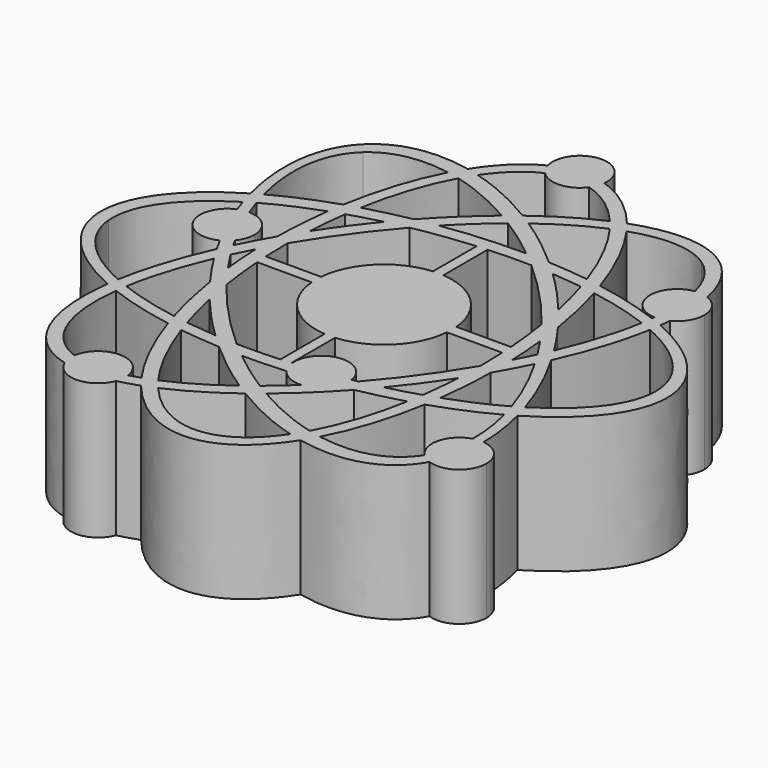
from build123d import *

# Parameters (mm, degrees)
F0_W     = 0.3843803424
F0_H     = 0.4350456002
F1_DEPTH = 5


# Not quite as in the source:
# - a feature names something its author has since deleted; it is built from what else it names


with BuildPart() as f1:
    # F0 (on Top) → F1 (new body)
    with BuildSketch(Plane.XY):
        with BuildLine():
            ThreePointArc((2.4905187876, -0.2175228001), (2.4976285722, -0.1088646659), (2.5, 0))
            ThreePointArc((2.5, 0), (2.4976285722, 0.1088646659), (2.4905187876, 0.2175228001))
            Line((2.4905187876, 0.2175228001), (0.1921901712, 0.2175228001))
            Line((0.1921901712, 0.2175228001), (0.1921901712, -0.2175228001))
            Line((0.1921901712, -0.2175228001), (2.4905187876, -0.2175228001))
        make_face()
        with BuildLine():
            ThreePointArc((2.4905187876, 0.2175228001), (2.4976285722, 0.1088646659), (2.5, 0))
            ThreePointArc((2.5, 0), (2.4976285722, -0.1088646659), (2.4905187876, -0.2175228001))
            Line((2.4905187876, -0.2175228001), (4.5236928473, -0.2175228001))
            add(Edge.make_bspline(
                [(4.5236928473, -0.2175228001), (4.5124932019, 0), (4.4965381449, 0.2175228001)],
                knots=[4.6512756828, 4.6512756828, 4.6512756828, 4.6971890264, 4.6971890264, 4.6971890264], degree=2, weights=[1, 0.9997365072, 1]))
            Line((4.4965381449, 0.2175228001), (2.4905187876, 0.2175228001))
        make_face()
        with BuildLine():
            Line((0.1921901712, 0.2175228001), (2.4905187876, 0.2175228001))
            ThreePointArc((2.4905187876, 0.2175228001), (1.7587574511, 1.7767307697), (0.1921901712, 2.4926016405))
            Line((0.1921901712, 2.4926016405), (0.1921901712, 0.2175228001))
        make_face()
        with BuildLine():
            ThreePointArc((0.1921901712, -2.4926016405), (1.7587574511, -1.7767307697), (2.4905187876, -0.2175228001))
            Line((2.4905187876, -0.2175228001), (0.1921901712, -0.2175228001))
            Line((0.1921901712, -0.2175228001), (0.1921901712, -2.4926016405))
        make_face()
        with BuildLine():
            Line((0.1921901712, 0.2175228001), (0.1921901712, 2.4926016405))
            ThreePointArc((0.1921901712, 2.4926016405), (0, 2.5), (-0.1921901712, 2.4926016405))
            Line((-0.1921901712, 2.4926016405), (-0.1921901712, 0.2175228001))
            Line((-0.1921901712, 0.2175228001), (0.1921901712, 0.2175228001))
        make_face()
        with BuildLine():
            ThreePointArc((-0.1921901712, 2.4926016405), (0, 2.5), (0.1921901712, 2.4926016405))
            Line((0.1921901712, 2.4926016405), (0.1921901712, 4.5264922249))
            add(Edge.make_bspline(
                [(0.1921901712, 4.5264922249), (0, 4.5149786018), (-0.1921901712, 4.4997461317)],
                knots=[4.6495476139, 4.6495476139, 4.6495476139, 4.6901378067, 4.6901378067, 4.6901378067], degree=2, weights=[1, 0.9997940616, 1]))
            Line((-0.1921901712, 4.4997461317), (-0.1921901712, 2.4926016405))
        make_face()
        Rectangle(F0_W, F0_H)
        with BuildLine():
            Line((4.8354491591, 0.2175228001), (4.4965381449, 0.2175228001))
            add(Edge.make_bspline(
                [(4.5236928473, -0.2175228001), (4.5124932019, 0), (4.4965381449, 0.2175228001)],
                knots=[4.6512756828, 4.6512756828, 4.6512756828, 4.6971890264, 4.6971890264, 4.6971890264], degree=2, weights=[1, 0.9997365072, 1]))
            Line((4.5236928473, -0.2175228001), (4.8354491591, -0.2175228001))
            Line((4.8354491591, -0.2175228001), (4.8354491591, 0.2175228001))
        make_face()
        with BuildLine():
            add(Edge.make_bspline(
                [(4.4965381449, 0.2175228001), (4.4354094642, 1.050918867), (4.3061600076, 1.8681745056)],
                knots=[4.6971890264, 4.6971890264, 4.6971890264, 4.872676185, 4.872676185, 4.872676185], degree=2, weights=[1, 0.9961530012, 1]))
            Line((4.4965381449, 0.2175228001), (4.8354491591, 0.2175228001))
            Line((4.8354491591, 0.2175228001), (4.8354491591, -0.2175228001))
            Line((4.8354491591, -0.2175228001), (4.5236928473, -0.2175228001))
            add(Edge.make_bspline(
                [(4.5499066856, -1.2491794731), (4.5503643102, -0.7355437777), (4.5236928473, -0.2175228001)],
                knots=[4.5420246596, 4.5420246596, 4.5420246596, 4.6512756828, 4.6512756828, 4.6512756828], degree=2, weights=[1, 0.9985083977, 1]))
            add(Edge.make_bspline(
                [(4.5499066856, -1.2491794731), (4.8032389245, -0.8217306737), (5.0297672297, -0.3896962987)],
                knots=[4.8827533011, 4.8827533011, 4.8827533011, 4.9884470587, 4.9884470587, 4.9884470587], degree=2, weights=[1, 0.9986039287, 1]))
            add(Edge.make_bspline(
                [(5.0297672297, -0.3896962987), (5.0027321886, 0.3203609711), (4.9252058483, 1.0271849194)],
                knots=[4.6348152583, 4.6348152583, 4.6348152583, 4.7770106723, 4.7770106723, 4.7770106723], degree=2, weights=[1, 0.9974736225, 1]))
            add(Edge.make_bspline(
                [(4.9252058483, 1.0271849194), (4.6301875685, 1.4522290012), (4.3061600076, 1.8681745056)],
                knots=[4.4401035362, 4.4401035362, 4.4401035362, 4.5521017758, 4.5521017758, 4.5521017758], degree=2, weights=[1, 0.998432459, 1]))
        make_face()
        with BuildLine():
            Line((0.1921901712, -4.4997461317), (0.1921901712, -2.4926016405))
            ThreePointArc((0.1921901712, -2.4926016405), (0, -2.5), (-0.1921901712, -2.4926016405))
            Line((-0.1921901712, -2.4926016405), (-0.1921901712, -4.5264922249))
            add(Edge.make_bspline(
                [(-0.1921901712, -4.5264922249), (0, -4.5149786018), (0.1921901712, -4.4997461317)],
                knots=[1.5079549603, 1.5079549603, 1.5079549603, 1.5485451531, 1.5485451531, 1.5485451531], degree=2, weights=[1, 0.9997940616, 1]))
        make_face()
        with BuildLine():
            ThreePointArc((-0.1921901712, -2.4926016405), (0, -2.5), (0.1921901712, -2.4926016405))
            Line((0.1921901712, -2.4926016405), (0.1921901712, -0.2175228001))
            Line((0.1921901712, -0.2175228001), (-0.1921901712, -0.2175228001))
            Line((-0.1921901712, -0.2175228001), (-0.1921901712, -2.4926016405))
        make_face()
        with BuildLine():
            Line((-0.1921901712, 0.2175228001), (-0.1921901712, 2.4926016405))
            ThreePointArc((-0.1921901712, 2.4926016405), (-1.7587574511, 1.7767307697), (-2.4905187876, 0.2175228001))
            Line((-2.4905187876, 0.2175228001), (-0.1921901712, 0.2175228001))
        make_face()
        with BuildLine():
            Line((0.1921901712, 4.7801313922), (0.1921901712, 4.5264922249))
            add(Edge.make_bspline(
                [(1.7753580031, 4.5575556434), (0.9907720796, 4.5743332311), (0.1921901712, 4.5264922249)],
                knots=[4.4812637681, 4.4812637681, 4.4812637681, 4.6495476139, 4.6495476139, 4.6495476139], degree=2, weights=[1, 0.9964621564, 1]))
            add(Edge.make_bspline(
                [(1.7753580031, 4.5575556434), (1.4925561491, 4.8063614912), (1.2048703246, 5.0394398721)],
                knots=[4.9435141927, 4.9435141927, 4.9435141927, 5.0244339682, 5.0244339682, 5.0244339682], degree=2, weights=[1, 0.9991816104, 1]))
            add(Edge.make_bspline(
                [(1.2048703246, 5.0394398721), (-0.3250854444, 5.0489630388), (-1.8398963463, 4.8232684303)],
                knots=[4.5547800949, 4.5547800949, 4.5547800949, 4.8612230288, 4.8612230288, 4.8612230288], degree=2, weights=[1, 0.9882845381, 1]))
            add(Edge.make_bspline(
                [(-1.8398963463, 4.8232684303), (-2.1316730534, 4.5196126683), (-2.4144520221, 4.1968797346)],
                knots=[1.2636379983, 1.2636379983, 1.2636379983, 1.3555504313, 1.3555504313, 1.3555504313], degree=2, weights=[1, 0.9989441989, 1]))
            add(Edge.make_bspline(
                [(-0.1921901712, 4.4997461317), (-1.3218736697, 4.4102104912), (-2.4144520221, 4.1968797346)],
                knots=[4.6901378067, 4.6901378067, 4.6901378067, 4.9276348759, 4.9276348759, 4.9276348759], degree=2, weights=[1, 0.992957674, 1]))
            Line((-0.1921901712, 4.4997461317), (-0.1921901712, 4.7801313922))
            Line((-0.1921901712, 4.7801313922), (0.1921901712, 4.7801313922))
        make_face()
        with BuildLine():
            add(Edge.make_bspline(
                [(0.1921901712, 4.5264922249), (0, 4.5149786018), (-0.1921901712, 4.4997461317)],
                knots=[4.6495476139, 4.6495476139, 4.6495476139, 4.6901378067, 4.6901378067, 4.6901378067], degree=2, weights=[1, 0.9997940616, 1]))
            Line((0.1921901712, 4.5264922249), (0.1921901712, 4.7801313922))
            Line((0.1921901712, 4.7801313922), (-0.1921901712, 4.7801313922))
            Line((-0.1921901712, 4.7801313922), (-0.1921901712, 4.4997461317))
        make_face()
        with BuildLine():
            Line((-0.1921901712, -0.2175228001), (-0.1921901712, 0.2175228001))
            Line((-0.1921901712, 0.2175228001), (-2.4905187876, 0.2175228001))
            ThreePointArc((-2.4905187876, 0.2175228001), (-2.5, 0), (-2.4905187876, -0.2175228001))
            Line((-2.4905187876, -0.2175228001), (-0.1921901712, -0.2175228001))
        make_face()
        with BuildLine():
            add(Edge.make_bspline(
                [(4.3061600076, 1.8681745056), (4.2255892515, 2.3776304558), (4.119680373, 2.8728292958)],
                knots=[4.872676185, 4.872676185, 4.872676185, 4.9822421902, 4.9822421902, 4.9822421902], degree=2, weights=[1, 0.9984997866, 1]))
            add(Edge.make_bspline(
                [(4.9252058483, 1.0271849194), (4.6301875685, 1.4522290012), (4.3061600076, 1.8681745056)],
                knots=[4.4401035362, 4.4401035362, 4.4401035362, 4.5521017758, 4.5521017758, 4.5521017758], degree=2, weights=[1, 0.998432459, 1]))
            add(Edge.make_bspline(
                [(4.9252058483, 1.0271849194), (4.8707697209, 1.5234905404), (4.7920342094, 2.0121957441)],
                knots=[4.7770106723, 4.7770106723, 4.7770106723, 4.8769403642, 4.8769403642, 4.8769403642], degree=2, weights=[1, 0.9987520167, 1]))
            add(Edge.make_bspline(
                [(4.7920342094, 2.0121957441), (4.46930502, 2.4498839961), (4.119680373, 2.8728292958)],
                knots=[4.5478375966, 4.5478375966, 4.5478375966, 4.6575997201, 4.6575997201, 4.6575997201], degree=2, weights=[1, 0.9984944125, 1]))
        make_face()
        with BuildLine():
            add(Edge.make_bspline(
                [(4.3061600076, 1.8681745056), (3.1602625104, 3.3391324429), (1.7753580031, 4.5575556434)],
                knots=[4.5521017758, 4.5521017758, 4.5521017758, 4.9435141927, 4.9435141927, 4.9435141927], degree=2, weights=[1, 0.9809105854, 1]))
            add(Edge.make_bspline(
                [(4.3061600076, 1.8681745056), (4.2255892515, 2.3776304558), (4.119680373, 2.8728292958)],
                knots=[4.872676185, 4.872676185, 4.872676185, 4.9822421902, 4.9822421902, 4.9822421902], degree=2, weights=[1, 0.9984997866, 1]))
            add(Edge.make_bspline(
                [(4.119680373, 2.8728292958), (3.3988038036, 3.7448826802), (2.5918169884, 4.5220577526)],
                knots=[4.6575997201, 4.6575997201, 4.6575997201, 4.8831797107, 4.8831797107, 4.8831797107], degree=2, weights=[1, 0.9936459489, 1]))
            add(Edge.make_bspline(
                [(2.5918169884, 4.5220577526), (2.187881526, 4.5487342392), (1.7753580031, 4.5575556434)],
                knots=[4.3926313072, 4.3926313072, 4.3926313072, 4.4812637681, 4.4812637681, 4.4812637681], degree=2, weights=[1, 0.9990181966, 1]))
        make_face()
        with BuildLine():
            ThreePointArc((-2.4905187876, -0.2175228001), (-1.7587574511, -1.7767307697), (-0.1921901712, -2.4926016405))
            Line((-0.1921901712, -2.4926016405), (-0.1921901712, -0.2175228001))
            Line((-0.1921901712, -0.2175228001), (-2.4905187876, -0.2175228001))
        make_face()
        with BuildLine():
            Line((0.1921901712, -4.7801313922), (0.1921901712, -4.4997461317))
            add(Edge.make_bspline(
                [(-0.1921901712, -4.5264922249), (0, -4.5149786018), (0.1921901712, -4.4997461317)],
                knots=[1.5079549603, 1.5079549603, 1.5079549603, 1.5485451531, 1.5485451531, 1.5485451531], degree=2, weights=[1, 0.9997940616, 1]))
            Line((-0.1921901712, -4.5264922249), (-0.1921901712, -4.7801313922))
            Line((-0.1921901712, -4.7801313922), (0.1921901712, -4.7801313922))
        make_face()
        with BuildLine():
            add(Edge.make_bspline(
                [(0.1921901712, -4.4997461317), (0.2034158574, -4.4988564144), (0.2146409717, -4.4979540498)],
                knots=[1.5485451531, 1.5485451531, 1.5485451531, 1.5509163207, 1.5509163207, 1.5509163207], degree=2, weights=[1, 0.9999992972, 1]))
            Line((0.1921901712, -4.4997461317), (0.1921901712, -4.7801313922))
            Line((0.1921901712, -4.7801313922), (-0.1921901712, -4.7801313922))
            Line((-0.1921901712, -4.7801313922), (-0.1921901712, -4.5264922249))
            add(Edge.make_bspline(
                [(-1.7753580031, -4.5575556434), (-0.9907720796, -4.5743332311), (-0.1921901712, -4.5264922249)],
                knots=[1.3396711145, 1.3396711145, 1.3396711145, 1.5079549603, 1.5079549603, 1.5079549603], degree=2, weights=[1, 0.9964621564, 1]))
            add(Edge.make_bspline(
                [(-1.7753580031, -4.5575556434), (-1.4925561491, -4.8063614912), (-1.2048703246, -5.0394398721)],
                knots=[1.8019215391, 1.8019215391, 1.8019215391, 1.8828413146, 1.8828413146, 1.8828413146], degree=2, weights=[1, 0.9991816104, 1]))
            add(Edge.make_bspline(
                [(-1.2048703246, -5.0394398721), (-0.4038678023, -5.0444256898), (0.4023806611, -4.9838881851)],
                knots=[1.4131874414, 1.4131874414, 1.4131874414, 1.574540911, 1.574540911, 1.574540911], degree=2, weights=[1, 0.996747397, 1]))
            ThreePointArc((0.4023806611, -4.9838881851), (0.2763123039, -4.7533609489), (0.2146409717, -4.4979540498))
        make_face()
        with BuildLine():
            add(Edge.make_bspline(
                [(4.5233594717, -2.2383499255), (4.5494616408, -1.7486956676), (4.5499066856, -1.2491794731)],
                knots=[4.4357711465, 4.4357711465, 4.4357711465, 4.5420246596, 4.5420246596, 4.5420246596], degree=2, weights=[1, 0.9985891058, 1]))
            add(Edge.make_bspline(
                [(2.4144520221, -4.1968797346), (3.6149021343, -2.8268174975), (4.5499066856, -1.2491794731)],
                knots=[4.4971430849, 4.4971430849, 4.4971430849, 4.8827533011, 4.8827533011, 4.8827533011], degree=2, weights=[1, 0.9814706027, 1]))
            add(Edge.make_bspline(
                [(2.4144520221, -4.1968797346), (2.8199560994, -4.1177032697), (3.2144229593, -4.0224102467)],
                knots=[1.7860422223, 1.7860422223, 1.7860422223, 1.8745467267, 1.8745467267, 1.8745467267], degree=2, weights=[1, 0.9990210289, 1]))
            add(Edge.make_bspline(
                [(3.2144229593, -4.0224102467), (3.9168714107, -3.1692016087), (4.5233594717, -2.2383499255)],
                knots=[4.569907423, 4.569907423, 4.569907423, 4.791717877, 4.791717877, 4.791717877], degree=2, weights=[1, 0.9938563164, 1]))
        make_face()
        with BuildLine():
            add(Edge.make_bspline(
                [(4.5499066856, -1.2491794731), (4.8032389245, -0.8217306737), (5.0297672297, -0.3896962987)],
                knots=[4.8827533011, 4.8827533011, 4.8827533011, 4.9884470587, 4.9884470587, 4.9884470587], degree=2, weights=[1, 0.9986039287, 1]))
            add(Edge.make_bspline(
                [(4.5233594717, -2.2383499255), (4.5494616408, -1.7486956676), (4.5499066856, -1.2491794731)],
                knots=[4.4357711465, 4.4357711465, 4.4357711465, 4.5420246596, 4.5420246596, 4.5420246596], degree=2, weights=[1, 0.9985891058, 1]))
            add(Edge.make_bspline(
                [(4.5233594717, -2.2383499255), (4.7947392542, -1.821830057), (5.042366833, -1.3962851974)],
                knots=[4.791717877, 4.791717877, 4.791717877, 4.8912959926, 4.8912959926, 4.8912959926], degree=2, weights=[1, 0.9987607809, 1]))
            add(Edge.make_bspline(
                [(5.042366833, -1.3962851974), (5.0490173215, -0.8952870816), (5.0297672297, -0.3896962987)],
                knots=[4.5334819682, 4.5334819682, 4.5334819682, 4.6348152583, 4.6348152583, 4.6348152583], degree=2, weights=[1, 0.9987167201, 1]))
        make_face()
        with BuildLine():
            ThreePointArc((-2.4905187876, -0.2175228001), (-2.5, 0), (-2.4905187876, 0.2175228001))
            Line((-2.4905187876, 0.2175228001), (-4.5236928473, 0.2175228001))
            add(Edge.make_bspline(
                [(-4.5236928473, 0.2175228001), (-4.5124932019, 0), (-4.4965381449, -0.2175228001)],
                knots=[1.5096830292, 1.5096830292, 1.5096830292, 1.5555963728, 1.5555963728, 1.5555963728], degree=2, weights=[1, 0.9997365072, 1]))
            Line((-4.4965381449, -0.2175228001), (-2.4905187876, -0.2175228001))
        make_face()
        with BuildLine():
            add(Edge.make_bspline(
                [(1.7753580031, 4.5575556434), (1.4925561491, 4.8063614912), (1.2048703246, 5.0394398721)],
                knots=[4.9435141927, 4.9435141927, 4.9435141927, 5.0244339682, 5.0244339682, 5.0244339682], degree=2, weights=[1, 0.9991816104, 1]))
            add(Edge.make_bspline(
                [(2.5918169884, 4.5220577526), (2.187881526, 4.5487342392), (1.7753580031, 4.5575556434)],
                knots=[4.3926313072, 4.3926313072, 4.3926313072, 4.4812637681, 4.4812637681, 4.4812637681], degree=2, weights=[1, 0.9990181966, 1]))
            add(Edge.make_bspline(
                [(2.5918169884, 4.5220577526), (2.3291205276, 4.7750496692), (2.060099324, 5.0150749057)],
                knots=[4.8831797107, 4.8831797107, 4.8831797107, 4.956891809, 4.956891809, 4.956891809], degree=2, weights=[1, 0.9993208927, 1]))
            add(Edge.make_bspline(
                [(2.060099324, 5.0150749057), (1.6355702489, 5.0367589925), (1.2048703246, 5.0394398721)],
                knots=[4.4678861517, 4.4678861517, 4.4678861517, 4.5547800949, 4.5547800949, 4.5547800949], degree=2, weights=[1, 0.9990563288, 1]))
        make_face()
        with BuildLine():
            add(Edge.make_bspline(
                [(4.9252058483, 1.0271849194), (4.8707697209, 1.5234905404), (4.7920342094, 2.0121957441)],
                knots=[4.7770106723, 4.7770106723, 4.7770106723, 4.8769403642, 4.8769403642, 4.8769403642], degree=2, weights=[1, 0.9987520167, 1]))
            add(Edge.make_bspline(
                [(5.3862832869, 0.3287868147), (5.1665909652, 0.6794121798), (4.9252058483, 1.0271849194)],
                knots=[4.3484344739, 4.3484344739, 4.3484344739, 4.4401035362, 4.4401035362, 4.4401035362], degree=2, weights=[1, 0.9989497818, 1]))
            add(Edge.make_bspline(
                [(5.3862832869, 0.3287868147), (5.5006657546, 0.573145213), (5.6052163125, 0.8164791695)],
                knots=[5.0763434868, 5.0763434868, 5.0763434868, 5.1361420873, 5.1361420873, 5.1361420873], degree=2, weights=[1, 0.9995530492, 1]))
            add(Edge.make_bspline(
                [(5.6052163125, 0.8164791695), (5.2271437791, 1.4220962019), (4.7920342094, 2.0121957441)],
                knots=[4.3999754692, 4.3999754692, 4.3999754692, 4.5478375966, 4.5478375966, 4.5478375966], degree=2, weights=[1, 0.9972683435, 1]))
        make_face()
        with BuildLine():
            add(Edge.make_bspline(
                [(4.119680373, 2.8728292958), (3.9491911042, 3.6699870915), (3.7176276788, 4.4103886148)],
                knots=[4.9822421902, 4.9822421902, 4.9822421902, 5.1583387825, 5.1583387825, 5.1583387825], degree=2, weights=[1, 0.9961262523, 1]))
            add(Edge.make_bspline(
                [(4.7920342094, 2.0121957441), (4.46930502, 2.4498839961), (4.119680373, 2.8728292958)],
                knots=[4.5478375966, 4.5478375966, 4.5478375966, 4.6575997201, 4.6575997201, 4.6575997201], degree=2, weights=[1, 0.9984944125, 1]))
            add(Edge.make_bspline(
                [(4.7920342094, 2.0121957441), (4.5977900484, 3.2178541644), (4.2656897661, 4.3270312557)],
                knots=[4.8769403642, 4.8769403642, 4.8769403642, 5.1224364643, 5.1224364643, 5.1224364643], degree=2, weights=[1, 0.9924759124, 1]))
            add(Edge.make_bspline(
                [(4.2656897661, 4.3270312557), (3.9957277913, 4.3731633675), (3.7176276788, 4.4103886148)],
                knots=[4.202604995, 4.202604995, 4.202604995, 4.2664391783, 4.2664391783, 4.2664391783], degree=2, weights=[1, 0.9994906929, 1]))
        make_face()
        with BuildLine():
            ThreePointArc((2.1970374676, -4.2380231848), (1.079108619, -3.4014612343), (0.2146409717, -4.4979540498))
            add(Edge.make_bspline(
                [(0.2146409717, -4.4979540498), (1.2194196531, -4.4171818909), (2.1970374676, -4.2380231848)],
                knots=[1.5509163207, 1.5509163207, 1.5509163207, 1.7623721378, 1.7623721378, 1.7623721378], degree=2, weights=[1, 0.9944160093, 1]))
        make_face()
        with BuildLine():
            add(Edge.make_bspline(
                [(0.2146409717, -4.4979540498), (1.2194196531, -4.4171818909), (2.1970374676, -4.2380231848)],
                knots=[1.5509163207, 1.5509163207, 1.5509163207, 1.7623721378, 1.7623721378, 1.7623721378], degree=2, weights=[1, 0.9944160093, 1]))
            ThreePointArc((0.2146409717, -4.4979540498), (0.2763123039, -4.7533609489), (0.4023806611, -4.9838881851))
            add(Edge.make_bspline(
                [(0.4023806611, -4.9838881851), (1.127059525, -4.9294753681), (1.8398963463, -4.8232684303)],
                knots=[1.574540911, 1.574540911, 1.574540911, 1.7196303752, 1.7196303752, 1.7196303752], degree=2, weights=[1, 0.9973697847, 1]))
            add(Edge.make_bspline(
                [(1.8398963463, -4.8232684303), (2.0259381119, -4.6296523782), (2.2084988867, -4.4280816025)],
                knots=[4.4052306518, 4.4052306518, 4.4052306518, 4.4638600665, 4.4638600665, 4.4638600665], degree=2, weights=[1, 0.9995703547, 1]))
            ThreePointArc((2.2084988867, -4.4280816025), (2.2089612121, -4.4105306808), (2.2091153364, -4.3929743473))
            ThreePointArc((2.2091153364, -4.3929743473), (2.2060912968, -4.3152637662), (2.1970374676, -4.2380231848))
        make_face()
        with BuildLine():
            add(Edge.make_bspline(
                [(2.2084988867, -4.4280816025), (2.3121157122, -4.3136751867), (2.4144520221, -4.1968797346)],
                knots=[4.4638600665, 4.4638600665, 4.4638600665, 4.4971430849, 4.4971430849, 4.4971430849], degree=2, weights=[1, 0.9998615333, 1]))
            add(Edge.make_bspline(
                [(2.1970374676, -4.2380231848), (2.3060677365, -4.2180422458), (2.4144520221, -4.1968797346)],
                knots=[1.7623721378, 1.7623721378, 1.7623721378, 1.7860422223, 1.7860422223, 1.7860422223], degree=2, weights=[1, 0.9999299667, 1]))
            ThreePointArc((2.1970374676, -4.2380231848), (2.2060912968, -4.3152637662), (2.2091153364, -4.3929743473))
            ThreePointArc((2.2091153364, -4.3929743473), (2.2089612121, -4.4105306808), (2.2084988867, -4.4280816025))
        make_face()
        with BuildLine():
            add(Edge.make_bspline(
                [(2.4144520221, -4.1968797346), (2.8199560994, -4.1177032697), (3.2144229593, -4.0224102467)],
                knots=[1.7860422223, 1.7860422223, 1.7860422223, 1.8745467267, 1.8745467267, 1.8745467267], degree=2, weights=[1, 0.9990210289, 1]))
            add(Edge.make_bspline(
                [(2.2084988867, -4.4280816025), (2.3121157122, -4.3136751867), (2.4144520221, -4.1968797346)],
                knots=[4.4638600665, 4.4638600665, 4.4638600665, 4.4971430849, 4.4971430849, 4.4971430849], degree=2, weights=[1, 0.9998615333, 1]))
            ThreePointArc((2.2084988867, -4.4280816025), (2.1861200899, -4.6061918691), (2.1322582162, -4.7774313977))
            add(Edge.make_bspline(
                [(2.1322582162, -4.7774313977), (2.388778222, -4.7352032819), (2.6419931732, -4.6864236555)],
                knots=[1.7495243308, 1.7495243308, 1.7495243308, 1.8021341121, 1.8021341121, 1.8021341121], degree=2, weights=[1, 0.9996540463, 1]))
            add(Edge.make_bspline(
                [(2.6419931732, -4.6864236555), (2.9339955454, -4.3630232717), (3.2144229593, -4.0224102467)],
                knots=[4.4810511951, 4.4810511951, 4.4810511951, 4.569907423, 4.569907423, 4.569907423], degree=2, weights=[1, 0.9990132337, 1]))
        make_face()
        with BuildLine():
            add(Edge.make_bspline(
                [(5.0297672297, -0.3896962987), (5.2180972419, -0.0305136395), (5.3862832869, 0.3287868147)],
                knots=[4.9884470587, 4.9884470587, 4.9884470587, 5.0763434868, 5.0763434868, 5.0763434868], degree=2, weights=[1, 0.9990344327, 1]))
            add(Edge.make_bspline(
                [(5.042366833, -1.3962851974), (5.0490173215, -0.8952870816), (5.0297672297, -0.3896962987)],
                knots=[4.5334819682, 4.5334819682, 4.5334819682, 4.6348152583, 4.6348152583, 4.6348152583], degree=2, weights=[1, 0.9987167201, 1]))
            add(Edge.make_bspline(
                [(5.042366833, -1.3962851974), (5.3941979055, -0.7916679529), (5.6922216134, -0.1791537852)],
                knots=[4.8912959926, 4.8912959926, 4.8912959926, 5.0326584517, 5.0326584517, 5.0326584517], degree=2, weights=[1, 0.9975031217, 1]))
            add(Edge.make_bspline(
                [(5.6922216134, -0.1791537852), (5.5453624641, 0.0748990403), (5.3862832869, 0.3287868147)],
                knots=[4.2820348052, 4.2820348052, 4.2820348052, 4.3484344739, 4.3484344739, 4.3484344739], degree=2, weights=[1, 0.9994489361, 1]))
        make_face()
        with BuildLine():
            add(Edge.make_bspline(
                [(4.5233594717, -2.2383499255), (4.7947392542, -1.821830057), (5.042366833, -1.3962851974)],
                knots=[4.791717877, 4.791717877, 4.791717877, 4.8912959926, 4.8912959926, 4.8912959926], degree=2, weights=[1, 0.9987607809, 1]))
            add(Edge.make_bspline(
                [(4.3847174109, -3.6959887742), (4.4834631125, -2.9867713322), (4.5233594717, -2.2383499255)],
                knots=[4.2735695243, 4.2735695243, 4.2735695243, 4.4357711465, 4.4357711465, 4.4357711465], degree=2, weights=[1, 0.9967131314, 1]))
            add(Edge.make_bspline(
                [(4.3847174109, -3.6959887742), (4.6424192179, -3.6138958848), (4.8913785024, -3.52499737)],
                knots=[2.0096157828, 2.0096157828, 2.0096157828, 2.0709961352, 2.0709961352, 2.0709961352], degree=2, weights=[1, 0.9995290935, 1]))
            add(Edge.make_bspline(
                [(4.8913785024, -3.52499737), (5.0278371398, -2.4908437284), (5.042366833, -1.3962851974)],
                knots=[4.3128037866, 4.3128037866, 4.3128037866, 4.5334819682, 4.5334819682, 4.5334819682], degree=2, weights=[1, 0.993918816, 1]))
        make_face()
        with BuildLine():
            Line((-4.8354491591, 0.2175228001), (-4.5236928473, 0.2175228001))
            add(Edge.make_bspline(
                [(-4.5499066856, 1.2491794731), (-4.5503643102, 0.7355437777), (-4.5236928473, 0.2175228001)],
                knots=[1.4004320061, 1.4004320061, 1.4004320061, 1.5096830292, 1.5096830292, 1.5096830292], degree=2, weights=[1, 0.9985083977, 1]))
            add(Edge.make_bspline(
                [(-4.5499066856, 1.2491794731), (-4.8032389245, 0.8217306737), (-5.0297672297, 0.3896962987)],
                knots=[1.7411606475, 1.7411606475, 1.7411606475, 1.8468544051, 1.8468544051, 1.8468544051], degree=2, weights=[1, 0.9986039287, 1]))
            add(Edge.make_bspline(
                [(-5.0297672297, 0.3896962987), (-5.0027321886, -0.3203609711), (-4.9252058483, -1.0271849194)],
                knots=[1.4932226047, 1.4932226047, 1.4932226047, 1.6354180188, 1.6354180188, 1.6354180188], degree=2, weights=[1, 0.9974736225, 1]))
            add(Edge.make_bspline(
                [(-4.9252058483, -1.0271849194), (-4.6301875685, -1.4522290012), (-4.3061600076, -1.8681745056)],
                knots=[1.2985108826, 1.2985108826, 1.2985108826, 1.4105091222, 1.4105091222, 1.4105091222], degree=2, weights=[1, 0.998432459, 1]))
            add(Edge.make_bspline(
                [(-4.4965381449, -0.2175228001), (-4.4354094642, -1.050918867), (-4.3061600076, -1.8681745056)],
                knots=[1.5555963728, 1.5555963728, 1.5555963728, 1.7310835314, 1.7310835314, 1.7310835314], degree=2, weights=[1, 0.9961530012, 1]))
            Line((-4.4965381449, -0.2175228001), (-4.8354491591, -0.2175228001))
            Line((-4.8354491591, -0.2175228001), (-4.8354491591, 0.2175228001))
        make_face()
        with BuildLine():
            add(Edge.make_bspline(
                [(-4.5236928473, 0.2175228001), (-4.5124932019, 0), (-4.4965381449, -0.2175228001)],
                knots=[1.5096830292, 1.5096830292, 1.5096830292, 1.5555963728, 1.5555963728, 1.5555963728], degree=2, weights=[1, 0.9997365072, 1]))
            Line((-4.5236928473, 0.2175228001), (-4.8354491591, 0.2175228001))
            Line((-4.8354491591, 0.2175228001), (-4.8354491591, -0.2175228001))
            Line((-4.8354491591, -0.2175228001), (-4.4965381449, -0.2175228001))
        make_face()
        with BuildLine():
            add(Edge.make_bspline(
                [(-2.4144520221, 4.1968797346), (-3.6149021343, 2.8268174975), (-4.5499066856, 1.2491794731)],
                knots=[1.3555504313, 1.3555504313, 1.3555504313, 1.7411606475, 1.7411606475, 1.7411606475], degree=2, weights=[1, 0.9814706027, 1]))
            add(Edge.make_bspline(
                [(-2.4144520221, 4.1968797346), (-2.8199560994, 4.1177032697), (-3.2144229593, 4.0224102467)],
                knots=[4.9276348759, 4.9276348759, 4.9276348759, 5.0161393803, 5.0161393803, 5.0161393803], degree=2, weights=[1, 0.9990210289, 1]))
            add(Edge.make_bspline(
                [(-3.2144229593, 4.0224102467), (-3.9168714107, 3.1692016087), (-4.5233594717, 2.2383499255)],
                knots=[1.4283147694, 1.4283147694, 1.4283147694, 1.6501252234, 1.6501252234, 1.6501252234], degree=2, weights=[1, 0.9938563164, 1]))
            add(Edge.make_bspline(
                [(-4.5233594717, 2.2383499255), (-4.5494616408, 1.7486956676), (-4.5499066856, 1.2491794731)],
                knots=[1.2941784929, 1.2941784929, 1.2941784929, 1.4004320061, 1.4004320061, 1.4004320061], degree=2, weights=[1, 0.9985891058, 1]))
        make_face()
        with BuildLine():
            add(Edge.make_bspline(
                [(-2.4144520221, 4.1968797346), (-2.8199560994, 4.1177032697), (-3.2144229593, 4.0224102467)],
                knots=[4.9276348759, 4.9276348759, 4.9276348759, 5.0161393803, 5.0161393803, 5.0161393803], degree=2, weights=[1, 0.9990210289, 1]))
            add(Edge.make_bspline(
                [(-1.8398963463, 4.8232684303), (-2.1316730534, 4.5196126683), (-2.4144520221, 4.1968797346)],
                knots=[1.2636379983, 1.2636379983, 1.2636379983, 1.3555504313, 1.3555504313, 1.3555504313], degree=2, weights=[1, 0.9989441989, 1]))
            add(Edge.make_bspline(
                [(-1.8398963463, 4.8232684303), (-2.2447625432, 4.7629466319), (-2.6419931732, 4.6864236555)],
                knots=[4.8612230288, 4.8612230288, 4.8612230288, 4.9437267657, 4.9437267657, 4.9437267657], degree=2, weights=[1, 0.9991492623, 1]))
            add(Edge.make_bspline(
                [(-2.6419931732, 4.6864236555), (-2.9339955454, 4.3630232717), (-3.2144229593, 4.0224102467)],
                knots=[1.3394585415, 1.3394585415, 1.3394585415, 1.4283147694, 1.4283147694, 1.4283147694], degree=2, weights=[1, 0.9990132337, 1]))
        make_face()
        with BuildLine():
            add(Edge.make_bspline(
                [(1.2048703246, 5.0394398721), (0.41901091, 5.6761304018), (-0.376972525, 6.1756759104)],
                knots=[5.0244339682, 5.0244339682, 5.0244339682, 5.2447048951, 5.2447048951, 5.2447048951], degree=2, weights=[1, 0.9939412179, 1]))
            add(Edge.make_bspline(
                [(2.060099324, 5.0150749057), (1.6355702489, 5.0367589925), (1.2048703246, 5.0394398721)],
                knots=[4.4678861517, 4.4678861517, 4.4678861517, 4.5547800949, 4.5547800949, 4.5547800949], degree=2, weights=[1, 0.9990563288, 1]))
            add(Edge.make_bspline(
                [(2.060099324, 5.0150749057), (1.0930842319, 5.8778620136), (0.0883271368, 6.5376983523)],
                knots=[4.956891809, 4.956891809, 4.956891809, 5.2204389149, 5.2204389149, 5.2204389149], degree=2, weights=[1, 0.9913304213, 1]))
            add(Edge.make_bspline(
                [(0.0883271368, 6.5376983523), (-0.1445020095, 6.364585069), (-0.376972525, 6.1756759104)],
                knots=[0.9680124583, 0.9680124583, 0.9680124583, 1.0384804121, 1.0384804121, 1.0384804121], degree=2, weights=[1, 0.9993793476, 1]))
        make_face()
        with BuildLine():
            add(Edge.make_bspline(
                [(2.5918169884, 4.5220577526), (2.3291205276, 4.7750496692), (2.060099324, 5.0150749057)],
                knots=[4.8831797107, 4.8831797107, 4.8831797107, 4.956891809, 4.956891809, 4.956891809], degree=2, weights=[1, 0.9993208927, 1]))
            add(Edge.make_bspline(
                [(3.7176276788, 4.4103886148), (3.1673150495, 4.484051022), (2.5918169884, 4.5220577526)],
                knots=[4.2664391783, 4.2664391783, 4.2664391783, 4.3926313072, 4.3926313072, 4.3926313072], degree=2, weights=[1, 0.9980101036, 1]))
            add(Edge.make_bspline(
                [(3.7176276788, 4.4103886148), (3.6438168927, 4.6463914221), (3.5642406579, 4.8750424517)],
                knots=[5.1583387825, 5.1583387825, 5.1583387825, 5.2146001861, 5.2146001861, 5.2146001861], degree=2, weights=[1, 0.9996043579, 1]))
            add(Edge.make_bspline(
                [(3.5642406579, 4.8750424517), (2.8296342072, 4.9757686197), (2.060099324, 5.0150749057)],
                knots=[4.3106012086, 4.3106012086, 4.3106012086, 4.4678861517, 4.4678861517, 4.4678861517], degree=2, weights=[1, 0.9969092742, 1]))
        make_face()
        with BuildLine():
            add(Edge.make_bspline(
                [(5.3862832869, 0.3287868147), (5.5006657546, 0.573145213), (5.6052163125, 0.8164791695)],
                knots=[5.0763434868, 5.0763434868, 5.0763434868, 5.1361420873, 5.1361420873, 5.1361420873], degree=2, weights=[1, 0.9995530492, 1]))
            add(Edge.make_bspline(
                [(5.6922216134, -0.1791537852), (5.5453624641, 0.0748990403), (5.3862832869, 0.3287868147)],
                knots=[4.2820348052, 4.2820348052, 4.2820348052, 4.3484344739, 4.3484344739, 4.3484344739], degree=2, weights=[1, 0.9994489361, 1]))
            add(Edge.make_bspline(
                [(5.6922216134, -0.1791537852), (5.8085776229, 0.0599872711), (5.9160641062, 0.2990367286)],
                knots=[5.0326584517, 5.0326584517, 5.0326584517, 5.0879279584, 5.0879279584, 5.0879279584], degree=2, weights=[1, 0.9996181845, 1]))
            add(Edge.make_bspline(
                [(5.9160641062, 0.2990367286), (5.766382808, 0.5583139601), (5.6052163125, 0.8164791695)],
                knots=[4.3368500024, 4.3368500024, 4.3368500024, 4.3999754692, 4.3999754692, 4.3999754692], degree=2, weights=[1, 0.9995019383, 1]))
        make_face()
        with BuildLine():
            add(Edge.make_bspline(
                [(3.7176276788, 4.4103886148), (3.6438168927, 4.6463914221), (3.5642406579, 4.8750424517)],
                knots=[5.1583387825, 5.1583387825, 5.1583387825, 5.2146001861, 5.2146001861, 5.2146001861], degree=2, weights=[1, 0.9996043579, 1]))
            add(Edge.make_bspline(
                [(4.2656897661, 4.3270312557), (3.9957277913, 4.3731633675), (3.7176276788, 4.4103886148)],
                knots=[4.202604995, 4.202604995, 4.202604995, 4.2664391783, 4.2664391783, 4.2664391783], degree=2, weights=[1, 0.9994906929, 1]))
            add(Edge.make_bspline(
                [(4.2656897661, 4.3270312557), (4.1955887626, 4.5611606173), (4.1198012539, 4.7891079944)],
                knots=[5.1224364643, 5.1224364643, 5.1224364643, 5.1745067944, 5.1745067944, 5.1745067944], degree=2, weights=[1, 0.9996611042, 1]))
            add(Edge.make_bspline(
                [(4.1198012539, 4.7891079944), (3.8455190421, 4.8364747346), (3.5642406579, 4.8750424517)],
                knots=[4.2502711664, 4.2502711664, 4.2502711664, 4.3106012086, 4.3106012086, 4.3106012086], degree=2, weights=[1, 0.9995450702, 1]))
        make_face()
        with BuildLine():
            add(Edge.make_bspline(
                [(-2.5918169884, -4.5220577526), (-2.187881526, -4.5487342392), (-1.7753580031, -4.5575556434)],
                knots=[1.2510386536, 1.2510386536, 1.2510386536, 1.3396711145, 1.3396711145, 1.3396711145], degree=2, weights=[1, 0.9990181966, 1]))
            add(Edge.make_bspline(
                [(-4.3061600076, -1.8681745056), (-3.1602625104, -3.3391324429), (-1.7753580031, -4.5575556434)],
                knots=[1.4105091222, 1.4105091222, 1.4105091222, 1.8019215391, 1.8019215391, 1.8019215391], degree=2, weights=[1, 0.9809105854, 1]))
            add(Edge.make_bspline(
                [(-4.3061600076, -1.8681745056), (-4.2255892515, -2.3776304558), (-4.119680373, -2.8728292958)],
                knots=[1.7310835314, 1.7310835314, 1.7310835314, 1.8406495366, 1.8406495366, 1.8406495366], degree=2, weights=[1, 0.9984997866, 1]))
            add(Edge.make_bspline(
                [(-4.119680373, -2.8728292958), (-3.3988038036, -3.7448826802), (-2.5918169884, -4.5220577526)],
                knots=[1.5160070666, 1.5160070666, 1.5160070666, 1.7415870571, 1.7415870571, 1.7415870571], degree=2, weights=[1, 0.9936459489, 1]))
        make_face()
        with BuildLine():
            add(Edge.make_bspline(
                [(-1.7753580031, -4.5575556434), (-1.4925561491, -4.8063614912), (-1.2048703246, -5.0394398721)],
                knots=[1.8019215391, 1.8019215391, 1.8019215391, 1.8828413146, 1.8828413146, 1.8828413146], degree=2, weights=[1, 0.9991816104, 1]))
            add(Edge.make_bspline(
                [(-2.5918169884, -4.5220577526), (-2.187881526, -4.5487342392), (-1.7753580031, -4.5575556434)],
                knots=[1.2510386536, 1.2510386536, 1.2510386536, 1.3396711145, 1.3396711145, 1.3396711145], degree=2, weights=[1, 0.9990181966, 1]))
            add(Edge.make_bspline(
                [(-2.5918169884, -4.5220577526), (-2.3291205276, -4.7750496692), (-2.060099324, -5.0150749057)],
                knots=[1.7415870571, 1.7415870571, 1.7415870571, 1.8152991555, 1.8152991555, 1.8152991555], degree=2, weights=[1, 0.9993208927, 1]))
            add(Edge.make_bspline(
                [(-2.060099324, -5.0150749057), (-1.6355702489, -5.0367589925), (-1.2048703246, -5.0394398721)],
                knots=[1.3262934981, 1.3262934981, 1.3262934981, 1.4131874414, 1.4131874414, 1.4131874414], degree=2, weights=[1, 0.9990563288, 1]))
        make_face()
        with BuildLine():
            add(Edge.make_bspline(
                [(0.4023806611, -4.9838881851), (1.127059525, -4.9294753681), (1.8398963463, -4.8232684303)],
                knots=[1.574540911, 1.574540911, 1.574540911, 1.7196303752, 1.7196303752, 1.7196303752], degree=2, weights=[1, 0.9973697847, 1]))
            ThreePointArc((0.4023806611, -4.9838881851), (0.7835605939, -5.2979070305), (1.2685358716, -5.3912073863))
            add(Edge.make_bspline(
                [(1.2685358716, -5.3912073863), (1.5572996146, -5.1173704742), (1.8398963463, -4.8232684303)],
                knots=[4.3162061181, 4.3162061181, 4.3162061181, 4.4052306518, 4.4052306518, 4.4052306518], degree=2, weights=[1, 0.9990094926, 1]))
        make_face()
        with BuildLine():
            add(Edge.make_bspline(
                [(3.2144229593, -4.0224102467), (3.8169525209, -3.8768546395), (4.3847174109, -3.6959887742)],
                knots=[1.8745467267, 1.8745467267, 1.8745467267, 2.0096157828, 2.0096157828, 2.0096157828], degree=2, weights=[1, 0.9977204104, 1]))
            add(Edge.make_bspline(
                [(2.6419931732, -4.6864236555), (2.9339955454, -4.3630232717), (3.2144229593, -4.0224102467)],
                knots=[4.4810511951, 4.4810511951, 4.4810511951, 4.569907423, 4.569907423, 4.569907423], degree=2, weights=[1, 0.9990132337, 1]))
            add(Edge.make_bspline(
                [(2.6419931732, -4.6864236555), (3.493449761, -4.5223980554), (4.2906415719, -4.2881247235)],
                knots=[1.8021341121, 1.8021341121, 1.8021341121, 1.9786202236, 1.9786202236, 1.9786202236], degree=2, weights=[1, 0.9961091073, 1]))
            add(Edge.make_bspline(
                [(4.2906415719, -4.2881247235), (4.3428347194, -3.9968012126), (4.3847174109, -3.6959887742)],
                knots=[4.2046482584, 4.2046482584, 4.2046482584, 4.2735695243, 4.2735695243, 4.2735695243], degree=2, weights=[1, 0.9994062911, 1]))
        make_face()
        with BuildLine():
            ThreePointArc((2.1322582162, -4.7774313977), (2.1861200899, -4.6061918691), (2.2084988867, -4.4280816025))
            add(Edge.make_bspline(
                [(1.8398963463, -4.8232684303), (2.0259381119, -4.6296523782), (2.2084988867, -4.4280816025)],
                knots=[4.4052306518, 4.4052306518, 4.4052306518, 4.4638600665, 4.4638600665, 4.4638600665], degree=2, weights=[1, 0.9995703547, 1]))
            add(Edge.make_bspline(
                [(1.8398963463, -4.8232684303), (1.9865210611, -4.8014225302), (2.1322582162, -4.7774313977)],
                knots=[1.7196303752, 1.7196303752, 1.7196303752, 1.7495243308, 1.7495243308, 1.7495243308], degree=2, weights=[1, 0.999888296, 1]))
        make_face()
        with BuildLine():
            add(Edge.make_bspline(
                [(4.3847174109, -3.6959887742), (4.6424192179, -3.6138958848), (4.8913785024, -3.52499737)],
                knots=[2.0096157828, 2.0096157828, 2.0096157828, 2.0709961352, 2.0709961352, 2.0709961352], degree=2, weights=[1, 0.9995290935, 1]))
            add(Edge.make_bspline(
                [(4.2906415719, -4.2881247235), (4.3428347194, -3.9968012126), (4.3847174109, -3.6959887742)],
                knots=[4.2046482584, 4.2046482584, 4.2046482584, 4.2735695243, 4.2735695243, 4.2735695243], degree=2, weights=[1, 0.9994062911, 1]))
            add(Edge.make_bspline(
                [(4.2906415719, -4.2881247235), (4.5491226101, -4.212164066), (4.8001227831, -4.1292766594)],
                knots=[1.9786202236, 1.9786202236, 1.9786202236, 2.0359772493, 2.0359772493, 2.0359772493], degree=2, weights=[1, 0.9995887996, 1]))
            add(Edge.make_bspline(
                [(4.8001227831, -4.1292766594), (4.8509669567, -3.8312568198), (4.8913785024, -3.52499737)],
                knots=[4.2472080579, 4.2472080579, 4.2472080579, 4.3128037866, 4.3128037866, 4.3128037866], degree=2, weights=[1, 0.9994621983, 1]))
        make_face()
        with BuildLine():
            add(Edge.make_bspline(
                [(-4.5499066856, 1.2491794731), (-4.8032389245, 0.8217306737), (-5.0297672297, 0.3896962987)],
                knots=[1.7411606475, 1.7411606475, 1.7411606475, 1.8468544051, 1.8468544051, 1.8468544051], degree=2, weights=[1, 0.9986039287, 1]))
            add(Edge.make_bspline(
                [(-4.5233594717, 2.2383499255), (-4.5494616408, 1.7486956676), (-4.5499066856, 1.2491794731)],
                knots=[1.2941784929, 1.2941784929, 1.2941784929, 1.4004320061, 1.4004320061, 1.4004320061], degree=2, weights=[1, 0.9985891058, 1]))
            add(Edge.make_bspline(
                [(-4.5233594717, 2.2383499255), (-4.7947392542, 1.821830057), (-5.042366833, 1.3962851974)],
                knots=[1.6501252234, 1.6501252234, 1.6501252234, 1.749703339, 1.749703339, 1.749703339], degree=2, weights=[1, 0.9987607809, 1]))
            add(Edge.make_bspline(
                [(-5.042366833, 1.3962851974), (-5.0490173215, 0.8952870816), (-5.0297672297, 0.3896962987)],
                knots=[1.3918893146, 1.3918893146, 1.3918893146, 1.4932226047, 1.4932226047, 1.4932226047], degree=2, weights=[1, 0.9987167201, 1]))
        make_face()
        with BuildLine():
            add(Edge.make_bspline(
                [(-3.2144229593, 4.0224102467), (-3.8169525209, 3.8768546395), (-4.3847174109, 3.6959887742)],
                knots=[5.0161393803, 5.0161393803, 5.0161393803, 5.1512084364, 5.1512084364, 5.1512084364], degree=2, weights=[1, 0.9977204104, 1]))
            add(Edge.make_bspline(
                [(-2.6419931732, 4.6864236555), (-2.9339955454, 4.3630232717), (-3.2144229593, 4.0224102467)],
                knots=[1.3394585415, 1.3394585415, 1.3394585415, 1.4283147694, 1.4283147694, 1.4283147694], degree=2, weights=[1, 0.9990132337, 1]))
            add(Edge.make_bspline(
                [(-2.6419931732, 4.6864236555), (-3.493449761, 4.5223980554), (-4.2906415719, 4.2881247235)],
                knots=[4.9437267657, 4.9437267657, 4.9437267657, 5.1202128772, 5.1202128772, 5.1202128772], degree=2, weights=[1, 0.9961091073, 1]))
            add(Edge.make_bspline(
                [(-4.2906415719, 4.2881247235), (-4.3428347194, 3.9968012126), (-4.3847174109, 3.6959887742)],
                knots=[1.0630556048, 1.0630556048, 1.0630556048, 1.1319768708, 1.1319768708, 1.1319768708], degree=2, weights=[1, 0.9994062911, 1]))
        make_face()
        with BuildLine():
            add(Edge.make_bspline(
                [(-1.8398963463, 4.8232684303), (-2.2447625432, 4.7629466319), (-2.6419931732, 4.6864236555)],
                knots=[4.8612230288, 4.8612230288, 4.8612230288, 4.9437267657, 4.9437267657, 4.9437267657], degree=2, weights=[1, 0.9991492623, 1]))
            add(Edge.make_bspline(
                [(-0.376972525, 6.1756759104), (-1.1226022733, 5.5697655737), (-1.8398963463, 4.8232684303)],
                knots=[1.0384804121, 1.0384804121, 1.0384804121, 1.2636379983, 1.2636379983, 1.2636379983], degree=2, weights=[1, 0.9936696978, 1]))
            add(Edge.make_bspline(
                [(-0.376972525, 6.1756759104), (-0.5967103845, 6.3135796103), (-0.8153371083, 6.4397267812)],
                knots=[5.2447048951, 5.2447048951, 5.2447048951, 5.305740625, 5.305740625, 5.305740625], degree=2, weights=[1, 0.9995343661, 1]))
            add(Edge.make_bspline(
                [(-0.8153371083, 6.4397267812), (-1.7598473168, 5.663423624), (-2.6419931732, 4.6864236555)],
                knots=[1.0724429349, 1.0724429349, 1.0724429349, 1.3394585415, 1.3394585415, 1.3394585415], degree=2, weights=[1, 0.9911010632, 1]))
        make_face()
        with BuildLine():
            add(Edge.make_bspline(
                [(-0.376972525, 6.1756759104), (-0.5967103845, 6.3135796103), (-0.8153371083, 6.4397267812)],
                knots=[5.2447048951, 5.2447048951, 5.2447048951, 5.305740625, 5.305740625, 5.305740625], degree=2, weights=[1, 0.9995343661, 1]))
            add(Edge.make_bspline(
                [(0.0883271368, 6.5376983523), (-0.1445020095, 6.364585069), (-0.376972525, 6.1756759104)],
                knots=[0.9680124583, 0.9680124583, 0.9680124583, 1.0384804121, 1.0384804121, 1.0384804121], degree=2, weights=[1, 0.9993793476, 1]))
            add(Edge.make_bspline(
                [(0.0883271368, 6.5376983523), (-0.1280783785, 6.6798145151), (-0.3442753147, 6.8110524147)],
                knots=[5.2204389149, 5.2204389149, 5.2204389149, 5.2775172812, 5.2775172812, 5.2775172812], degree=2, weights=[1, 0.9995927852, 1]))
            add(Edge.make_bspline(
                [(-0.3442753147, 6.8110524147), (-0.5804530149, 6.6327805582), (-0.8153371083, 6.4397267812)],
                knots=[1.005668026, 1.005668026, 1.005668026, 1.0724429349, 1.0724429349, 1.0724429349], degree=2, weights=[1, 0.9994426907, 1]))
        make_face()
        with BuildLine():
            add(Edge.make_bspline(
                [(5.6922216134, -0.1791537852), (5.8085776229, 0.0599872711), (5.9160641062, 0.2990367286)],
                knots=[5.0326584517, 5.0326584517, 5.0326584517, 5.0879279584, 5.0879279584, 5.0879279584], degree=2, weights=[1, 0.9996181845, 1]))
            add(Edge.make_bspline(
                [(6.8208068866, -2.6569887548), (6.4312972876, -1.4576867482), (5.6922216134, -0.1791537852)],
                knots=[3.9508141753, 3.9508141753, 3.9508141753, 4.2820348052, 4.2820348052, 4.2820348052], degree=2, weights=[1, 0.986317926, 1]))
            add(Edge.make_bspline(
                [(6.8208068866, -2.6569887548), (6.9945786489, -2.558908502), (7.1585711198, -2.4572505768)],
                knots=[2.3323711319, 2.3323711319, 2.3323711319, 2.3852568644, 2.3852568644, 2.3852568644], degree=2, weights=[1, 0.9996504078, 1]))
            add(Edge.make_bspline(
                [(7.1585711198, -2.4572505768), (6.7300342146, -1.1109184149), (5.9160641062, 0.2990367286)],
                knots=[3.9967742018, 3.9967742018, 3.9967742018, 4.3368500024, 4.3368500024, 4.3368500024], degree=2, weights=[1, 0.9855783541, 1]))
        make_face()
        with BuildLine():
            add(Edge.make_bspline(
                [(5.6052163125, 0.8164791695), (6.2677469531, 2.3584719164), (6.4956120061, 3.7369056381)],
                knots=[5.1361420873, 5.1361420873, 5.1361420873, 5.510752012, 5.510752012, 5.510752012], degree=2, weights=[1, 0.9825096501, 1]))
            add(Edge.make_bspline(
                [(5.9160641062, 0.2990367286), (5.766382808, 0.5583139601), (5.6052163125, 0.8164791695)],
                knots=[4.3368500024, 4.3368500024, 4.3368500024, 4.3999754692, 4.3999754692, 4.3999754692], degree=2, weights=[1, 0.9995019383, 1]))
            add(Edge.make_bspline(
                [(5.9160641062, 0.2990367286), (6.6806162303, 1.9993972287), (6.9478748431, 3.550926059)],
                knots=[5.0879279584, 5.0879279584, 5.0879279584, 5.4762076545, 5.4762076545, 5.4762076545], degree=2, weights=[1, 0.9812139753, 1]))
            add(Edge.make_bspline(
                [(6.9478748431, 3.550926059), (6.7294841299, 3.6481121526), (6.4956120061, 3.7369056381)],
                knots=[3.8461817573, 3.8461817573, 3.8461817573, 3.9140259488, 3.9140259488, 3.9140259488], degree=2, weights=[1, 0.9994247009, 1]))
        make_face()
        with BuildLine():
            add(Edge.make_bspline(
                [(4.2656897661, 4.3270312557), (4.1955887626, 4.5611606173), (4.1198012539, 4.7891079944)],
                knots=[5.1224364643, 5.1224364643, 5.1224364643, 5.1745067944, 5.1745067944, 5.1745067944], degree=2, weights=[1, 0.9996611042, 1]))
            add(Edge.make_bspline(
                [(6.4956120061, 3.7369056381), (5.4942465408, 4.1170908801), (4.2656897661, 4.3270312557)],
                knots=[3.9140259488, 3.9140259488, 3.9140259488, 4.202604995, 4.202604995, 4.202604995], degree=2, weights=[1, 0.9896083147, 1]))
            add(Edge.make_bspline(
                [(6.4956120061, 3.7369056381), (6.5292822637, 3.9405885545), (6.5527188245, 4.1380951736)],
                knots=[5.510752012, 5.510752012, 5.510752012, 5.5667477911, 5.5667477911, 5.5667477911], degree=2, weights=[1, 0.9996080847, 1]))
            add(Edge.make_bspline(
                [(6.5527188245, 4.1380951736), (5.4506442627, 4.5592801299), (4.1198012539, 4.7891079944)],
                knots=[3.9595210193, 3.9595210193, 3.9595210193, 4.2502711664, 4.2502711664, 4.2502711664], degree=2, weights=[1, 0.989451641, 1]))
        make_face()
        with BuildLine():
            add(Edge.make_bspline(
                [(3.5642406579, 4.8750424517), (2.9696241235, 6.5835887677), (2.1235631204, 7.7346884466)],
                knots=[5.2146001861, 5.2146001861, 5.2146001861, 5.6290752415, 5.6290752415, 5.6290752415], degree=2, weights=[1, 0.9786030469, 1]))
            add(Edge.make_bspline(
                [(4.1198012539, 4.7891079944), (3.8455190421, 4.8364747346), (3.5642406579, 4.8750424517)],
                knots=[4.2502711664, 4.2502711664, 4.2502711664, 4.3106012086, 4.3106012086, 4.3106012086], degree=2, weights=[1, 0.9995450702, 1]))
            add(Edge.make_bspline(
                [(4.1198012539, 4.7891079944), (3.5064173549, 6.6339931649), (2.594766926, 7.9145706904)],
                knots=[5.1745067944, 5.1745067944, 5.1745067944, 5.5899514307, 5.5899514307, 5.5899514307], degree=2, weights=[1, 0.9785031827, 1]))
            add(Edge.make_bspline(
                [(2.594766926, 7.9145706904), (2.362610327, 7.8360565885), (2.1235631204, 7.7346884466)],
                knots=[0.5777171095, 0.5777171095, 0.5777171095, 0.6541100657, 0.6541100657, 0.6541100657], degree=2, weights=[1, 0.9992706032, 1]))
        make_face()
        with BuildLine():
            add(Edge.make_bspline(
                [(-4.3061600076, -1.8681745056), (-4.2255892515, -2.3776304558), (-4.119680373, -2.8728292958)],
                knots=[1.7310835314, 1.7310835314, 1.7310835314, 1.8406495366, 1.8406495366, 1.8406495366], degree=2, weights=[1, 0.9984997866, 1]))
            add(Edge.make_bspline(
                [(-4.9252058483, -1.0271849194), (-4.6301875685, -1.4522290012), (-4.3061600076, -1.8681745056)],
                knots=[1.2985108826, 1.2985108826, 1.2985108826, 1.4105091222, 1.4105091222, 1.4105091222], degree=2, weights=[1, 0.998432459, 1]))
            add(Edge.make_bspline(
                [(-4.9252058483, -1.0271849194), (-4.8707697209, -1.5234905404), (-4.7920342094, -2.0121957441)],
                knots=[1.6354180188, 1.6354180188, 1.6354180188, 1.7353477106, 1.7353477106, 1.7353477106], degree=2, weights=[1, 0.9987520167, 1]))
            add(Edge.make_bspline(
                [(-4.7920342094, -2.0121957441), (-4.46930502, -2.4498839961), (-4.119680373, -2.8728292958)],
                knots=[1.406244943, 1.406244943, 1.406244943, 1.5160070666, 1.5160070666, 1.5160070666], degree=2, weights=[1, 0.9984944125, 1]))
        make_face()
        with BuildLine():
            add(Edge.make_bspline(
                [(-1.2048703246, -5.0394398721), (-0.41901091, -5.6761304018), (0.376972525, -6.1756759104)],
                knots=[1.8828413146, 1.8828413146, 1.8828413146, 2.1031122415, 2.1031122415, 2.1031122415], degree=2, weights=[1, 0.9939412179, 1]))
            add(Edge.make_bspline(
                [(-2.060099324, -5.0150749057), (-1.6355702489, -5.0367589925), (-1.2048703246, -5.0394398721)],
                knots=[1.3262934981, 1.3262934981, 1.3262934981, 1.4131874414, 1.4131874414, 1.4131874414], degree=2, weights=[1, 0.9990563288, 1]))
            add(Edge.make_bspline(
                [(-2.060099324, -5.0150749057), (-1.0930842319, -5.8778620136), (-0.0883271368, -6.5376983523)],
                knots=[1.8152991555, 1.8152991555, 1.8152991555, 2.0788462613, 2.0788462613, 2.0788462613], degree=2, weights=[1, 0.9913304213, 1]))
            add(Edge.make_bspline(
                [(-0.0883271368, -6.5376983523), (0.1445020095, -6.364585069), (0.376972525, -6.1756759104)],
                knots=[4.1096051119, 4.1096051119, 4.1096051119, 4.1800730657, 4.1800730657, 4.1800730657], degree=2, weights=[1, 0.9993793476, 1]))
        make_face()
        with BuildLine():
            add(Edge.make_bspline(
                [(-2.5918169884, -4.5220577526), (-2.3291205276, -4.7750496692), (-2.060099324, -5.0150749057)],
                knots=[1.7415870571, 1.7415870571, 1.7415870571, 1.8152991555, 1.8152991555, 1.8152991555], degree=2, weights=[1, 0.9993208927, 1]))
            add(Edge.make_bspline(
                [(-3.7176276788, -4.4103886148), (-3.1673150495, -4.484051022), (-2.5918169884, -4.5220577526)],
                knots=[1.1248465247, 1.1248465247, 1.1248465247, 1.2510386536, 1.2510386536, 1.2510386536], degree=2, weights=[1, 0.9980101036, 1]))
            add(Edge.make_bspline(
                [(-3.7176276788, -4.4103886148), (-3.6438168927, -4.6463914221), (-3.5642406579, -4.8750424517)],
                knots=[2.0167461289, 2.0167461289, 2.0167461289, 2.0730075325, 2.0730075325, 2.0730075325], degree=2, weights=[1, 0.9996043579, 1]))
            add(Edge.make_bspline(
                [(-3.5642406579, -4.8750424517), (-2.8296342072, -4.9757686197), (-2.060099324, -5.0150749057)],
                knots=[1.169008555, 1.169008555, 1.169008555, 1.3262934981, 1.3262934981, 1.3262934981], degree=2, weights=[1, 0.9969092742, 1]))
        make_face()
        with BuildLine():
            add(Edge.make_bspline(
                [(1.8398963463, -4.8232684303), (1.9865210611, -4.8014225302), (2.1322582162, -4.7774313977)],
                knots=[1.7196303752, 1.7196303752, 1.7196303752, 1.7495243308, 1.7495243308, 1.7495243308], degree=2, weights=[1, 0.999888296, 1]))
            add(Edge.make_bspline(
                [(1.2685358716, -5.3912073863), (1.5572996146, -5.1173704742), (1.8398963463, -4.8232684303)],
                knots=[4.3162061181, 4.3162061181, 4.3162061181, 4.4052306518, 4.4052306518, 4.4052306518], degree=2, weights=[1, 0.9990094926, 1]))
            ThreePointArc((1.2685358716, -5.3912073863), (1.7883717193, -5.2081197595), (2.1322582162, -4.7774313977))
        make_face()
        with BuildLine():
            ThreePointArc((2.1322582162, -4.7774313977), (1.7883717193, -5.2081197595), (1.2685358716, -5.3912073863))
            add(Edge.make_bspline(
                [(0.376972525, -6.1756759104), (0.826577866, -5.8103196137), (1.2685358716, -5.3912073863)],
                knots=[4.1800730657, 4.1800730657, 4.1800730657, 4.3162061181, 4.3162061181, 4.3162061181], degree=2, weights=[1, 0.9976843682, 1]))
            add(Edge.make_bspline(
                [(0.376972525, -6.1756759104), (0.5967103845, -6.3135796103), (0.8153371083, -6.4397267812)],
                knots=[2.1031122415, 2.1031122415, 2.1031122415, 2.1641479714, 2.1641479714, 2.1641479714], degree=2, weights=[1, 0.9995343661, 1]))
            add(Edge.make_bspline(
                [(0.8153371083, -6.4397267812), (1.7598473168, -5.663423624), (2.6419931732, -4.6864236555)],
                knots=[4.2140355885, 4.2140355885, 4.2140355885, 4.4810511951, 4.4810511951, 4.4810511951], degree=2, weights=[1, 0.9911010632, 1]))
            add(Edge.make_bspline(
                [(2.1322582162, -4.7774313977), (2.388778222, -4.7352032819), (2.6419931732, -4.6864236555)],
                knots=[1.7495243308, 1.7495243308, 1.7495243308, 1.8021341121, 1.8021341121, 1.8021341121], degree=2, weights=[1, 0.9996540463, 1]))
        make_face()
        with BuildLine():
            add(Edge.make_bspline(
                [(4.8913785024, -3.52499737), (5.9572601378, -3.1443917843), (6.8208068866, -2.6569887548)],
                knots=[2.0709961352, 2.0709961352, 2.0709961352, 2.3323711319, 2.3323711319, 2.3323711319], degree=2, weights=[1, 0.9914725361, 1]))
            add(Edge.make_bspline(
                [(4.8001227831, -4.1292766594), (4.8509669567, -3.8312568198), (4.8913785024, -3.52499737)],
                knots=[4.2472080579, 4.2472080579, 4.2472080579, 4.3128037866, 4.3128037866, 4.3128037866], degree=2, weights=[1, 0.9994621983, 1]))
            add(Edge.make_bspline(
                [(4.8001227831, -4.1292766594), (6.0005166906, -3.7328723993), (6.9792076076, -3.1985485205)],
                knots=[2.0359772493, 2.0359772493, 2.0359772493, 2.3086569246, 2.3086569246, 2.3086569246], degree=2, weights=[1, 0.9907201127, 1]))
            add(Edge.make_bspline(
                [(6.9792076076, -3.1985485205), (6.9101483801, -2.9320716608), (6.8208068866, -2.6569887548)],
                knots=[3.8741776453, 3.8741776453, 3.8741776453, 3.9508141753, 3.9508141753, 3.9508141753], degree=2, weights=[1, 0.9992659451, 1]))
        make_face()
        with BuildLine():
            add(Edge.make_bspline(
                [(4.2906415719, -4.2881247235), (4.5491226101, -4.212164066), (4.8001227831, -4.1292766594)],
                knots=[1.9786202236, 1.9786202236, 1.9786202236, 2.0359772493, 2.0359772493, 2.0359772493], degree=2, weights=[1, 0.9995887996, 1]))
            add(Edge.make_bspline(
                [(3.2413476203, -7.4713371001), (3.953143182, -6.1719202119), (4.2906415719, -4.2881247235)],
                knots=[3.7659763834, 3.7659763834, 3.7659763834, 4.2046482584, 4.2046482584, 4.2046482584], degree=2, weights=[1, 0.9760421523, 1]))
            add(Edge.make_bspline(
                [(3.2413476203, -7.4713371001), (3.4755473495, -7.5313860958), (3.7005606087, -7.5715283415)],
                knots=[2.5172089238, 2.5172089238, 2.5172089238, 2.589932199, 2.589932199, 2.589932199], degree=2, weights=[1, 0.9993389885, 1]))
            add(Edge.make_bspline(
                [(3.7005606087, -7.5715283415), (4.457775145, -6.1359252315), (4.8001227831, -4.1292766594)],
                knots=[3.8123600682, 3.8123600682, 3.8123600682, 4.2472080579, 4.2472080579, 4.2472080579], degree=2, weights=[1, 0.9764563714, 1]))
        make_face()
        with BuildLine():
            add(Edge.make_bspline(
                [(-5.0297672297, 0.3896962987), (-5.2180972419, 0.0305136395), (-5.3862832869, -0.3287868147)],
                knots=[1.8468544051, 1.8468544051, 1.8468544051, 1.9347508332, 1.9347508332, 1.9347508332], degree=2, weights=[1, 0.9990344327, 1]))
            add(Edge.make_bspline(
                [(-5.042366833, 1.3962851974), (-5.0490173215, 0.8952870816), (-5.0297672297, 0.3896962987)],
                knots=[1.3918893146, 1.3918893146, 1.3918893146, 1.4932226047, 1.4932226047, 1.4932226047], degree=2, weights=[1, 0.9987167201, 1]))
            add(Edge.make_bspline(
                [(-5.042366833, 1.3962851974), (-5.3941979055, 0.7916679529), (-5.6922216134, 0.1791537852)],
                knots=[1.749703339, 1.749703339, 1.749703339, 1.8910657981, 1.8910657981, 1.8910657981], degree=2, weights=[1, 0.9975031217, 1]))
            add(Edge.make_bspline(
                [(-5.6922216134, 0.1791537852), (-5.5453624641, -0.0748990403), (-5.3862832869, -0.3287868147)],
                knots=[1.1404421516, 1.1404421516, 1.1404421516, 1.2068418204, 1.2068418204, 1.2068418204], degree=2, weights=[1, 0.9994489361, 1]))
        make_face()
        with BuildLine():
            add(Edge.make_bspline(
                [(-4.5233594717, 2.2383499255), (-4.7947392542, 1.821830057), (-5.042366833, 1.3962851974)],
                knots=[1.6501252234, 1.6501252234, 1.6501252234, 1.749703339, 1.749703339, 1.749703339], degree=2, weights=[1, 0.9987607809, 1]))
            add(Edge.make_bspline(
                [(-4.3847174109, 3.6959887742), (-4.4834631125, 2.9867713322), (-4.5233594717, 2.2383499255)],
                knots=[1.1319768708, 1.1319768708, 1.1319768708, 1.2941784929, 1.2941784929, 1.2941784929], degree=2, weights=[1, 0.9967131314, 1]))
            add(Edge.make_bspline(
                [(-4.3847174109, 3.6959887742), (-4.6424192179, 3.6138958848), (-4.8913785024, 3.52499737)],
                knots=[5.1512084364, 5.1512084364, 5.1512084364, 5.2125887888, 5.2125887888, 5.2125887888], degree=2, weights=[1, 0.9995290935, 1]))
            add(Edge.make_bspline(
                [(-4.8913785024, 3.52499737), (-5.0278371398, 2.4908437284), (-5.042366833, 1.3962851974)],
                knots=[1.171211133, 1.171211133, 1.171211133, 1.3918893146, 1.3918893146, 1.3918893146], degree=2, weights=[1, 0.993918816, 1]))
        make_face()
        with BuildLine():
            add(Edge.make_bspline(
                [(-4.3847174109, 3.6959887742), (-4.6424192179, 3.6138958848), (-4.8913785024, 3.52499737)],
                knots=[5.1512084364, 5.1512084364, 5.1512084364, 5.2125887888, 5.2125887888, 5.2125887888], degree=2, weights=[1, 0.9995290935, 1]))
            add(Edge.make_bspline(
                [(-4.2906415719, 4.2881247235), (-4.3428347194, 3.9968012126), (-4.3847174109, 3.6959887742)],
                knots=[1.0630556048, 1.0630556048, 1.0630556048, 1.1319768708, 1.1319768708, 1.1319768708], degree=2, weights=[1, 0.9994062911, 1]))
            add(Edge.make_bspline(
                [(-4.2906415719, 4.2881247235), (-4.5491226101, 4.212164066), (-4.8001227831, 4.1292766594)],
                knots=[5.1202128772, 5.1202128772, 5.1202128772, 5.1775699029, 5.1775699029, 5.1775699029], degree=2, weights=[1, 0.9995887996, 1]))
            add(Edge.make_bspline(
                [(-4.8001227831, 4.1292766594), (-4.8509669567, 3.8312568198), (-4.8913785024, 3.52499737)],
                knots=[1.1056154043, 1.1056154043, 1.1056154043, 1.171211133, 1.171211133, 1.171211133], degree=2, weights=[1, 0.9994621983, 1]))
        make_face()
        with BuildLine():
            add(Edge.make_bspline(
                [(0.0883271368, 6.5376983523), (-0.1280783785, 6.6798145151), (-0.3442753147, 6.8110524147)],
                knots=[5.2204389149, 5.2204389149, 5.2204389149, 5.2775172812, 5.2775172812, 5.2775172812], degree=2, weights=[1, 0.9995927852, 1]))
            add(Edge.make_bspline(
                [(2.1235631204, 7.7346884466), (1.1336423563, 7.3149118264), (0.0883271368, 6.5376983523)],
                knots=[0.6541100657, 0.6541100657, 0.6541100657, 0.9680124583, 0.9680124583, 0.9680124583], degree=2, weights=[1, 0.9877084243, 1]))
            add(Edge.make_bspline(
                [(2.1235631204, 7.7346884466), (1.9768866304, 7.9342476508), (1.8249638751, 8.112750934)],
                knots=[5.6290752415, 5.6290752415, 5.6290752415, 5.701944665, 5.701944665, 5.701944665], degree=2, weights=[1, 0.9993363293, 1]))
            add(Edge.make_bspline(
                [(1.8249638751, 8.112750934), (0.7583453214, 7.6433334797), (-0.3442753147, 6.8110524147)],
                knots=[0.6962977279, 0.6962977279, 0.6962977279, 1.005668026, 1.005668026, 1.005668026], degree=2, weights=[1, 0.9880600885, 1]))
        make_face()
        with BuildLine():
            add(Edge.make_bspline(
                [(-0.8153371083, 6.4397267812), (-2.0928883815, 7.1768712432), (-3.2413476203, 7.4713371001)],
                knots=[5.305740625, 5.305740625, 5.305740625, 5.6588015774, 5.6588015774, 5.6588015774], degree=2, weights=[1, 0.9844589174, 1]))
            add(Edge.make_bspline(
                [(-0.3442753147, 6.8110524147), (-0.5804530149, 6.6327805582), (-0.8153371083, 6.4397267812)],
                knots=[1.005668026, 1.005668026, 1.005668026, 1.0724429349, 1.0724429349, 1.0724429349], degree=2, weights=[1, 0.9994426907, 1]))
            add(Edge.make_bspline(
                [(-0.3442753147, 6.8110524147), (-1.690108764, 7.6280129057), (-2.9324650451, 7.9779471368)],
                knots=[5.2775172812, 5.2775172812, 5.2775172812, 5.6292567073, 5.6292567073, 5.6292567073], degree=2, weights=[1, 0.9845747424, 1]))
            add(Edge.make_bspline(
                [(-2.9324650451, 7.9779471368), (-3.0935226365, 7.7411986879), (-3.2413476203, 7.4713371001)],
                knots=[0.5318572593, 0.5318572593, 0.5318572593, 0.6243837298, 0.6243837298, 0.6243837298], degree=2, weights=[1, 0.9989300474, 1]))
        make_face()
        with BuildLine():
            add(Edge.make_bspline(
                [(6.8208068866, -2.6569887548), (6.9945786489, -2.558908502), (7.1585711198, -2.4572505768)],
                knots=[2.3323711319, 2.3323711319, 2.3323711319, 2.3852568644, 2.3852568644, 2.3852568644], degree=2, weights=[1, 0.9996504078, 1]))
            add(Edge.make_bspline(
                [(6.9792076076, -3.1985485205), (6.9101483801, -2.9320716608), (6.8208068866, -2.6569887548)],
                knots=[3.8741776453, 3.8741776453, 3.8741776453, 3.9508141753, 3.9508141753, 3.9508141753], degree=2, weights=[1, 0.9992659451, 1]))
            add(Edge.make_bspline(
                [(6.9792076076, -3.1985485205), (7.1524129204, -3.1039857399), (7.3171905367, -3.0057655292)],
                knots=[2.3086569246, 2.3086569246, 2.3086569246, 2.3572065411, 2.3572065411, 2.3572065411], degree=2, weights=[1, 0.9997053813, 1]))
            add(Edge.make_bspline(
                [(7.3171905367, -3.0057655292), (7.2469574626, -2.7349334893), (7.1585711198, -2.4572505768)],
                knots=[3.9259787661, 3.9259787661, 3.9259787661, 3.9967742018, 3.9967742018, 3.9967742018], degree=2, weights=[1, 0.9993735662, 1]))
        make_face()
        with BuildLine():
            add(Edge.make_bspline(
                [(6.4956120061, 3.7369056381), (6.5292822637, 3.9405885545), (6.5527188245, 4.1380951736)],
                knots=[5.510752012, 5.510752012, 5.510752012, 5.5667477911, 5.5667477911, 5.5667477911], degree=2, weights=[1, 0.9996080847, 1]))
            add(Edge.make_bspline(
                [(6.9478748431, 3.550926059), (6.7294841299, 3.6481121526), (6.4956120061, 3.7369056381)],
                knots=[3.8461817573, 3.8461817573, 3.8461817573, 3.9140259488, 3.9140259488, 3.9140259488], degree=2, weights=[1, 0.9994247009, 1]))
            add(Edge.make_bspline(
                [(6.9478748431, 3.550926059), (6.9827621157, 3.7534587625), (7.0084558923, 3.9510496667)],
                knots=[5.4762076545, 5.4762076545, 5.4762076545, 5.5275279777, 5.5275279777, 5.5275279777], degree=2, weights=[1, 0.9996707961, 1]))
            add(Edge.make_bspline(
                [(7.0084558923, 3.9510496667), (6.7871648492, 4.0484958469), (6.5527188245, 4.1380951736)],
                knots=[3.8972499831, 3.8972499831, 3.8972499831, 3.9595210193, 3.9595210193, 3.9595210193], degree=2, weights=[1, 0.9995153289, 1]))
        make_face()
        with BuildLine():
            add(Edge.make_bspline(
                [(2.1235631204, 7.7346884466), (1.9768866304, 7.9342476508), (1.8249638751, 8.112750934)],
                knots=[5.6290752415, 5.6290752415, 5.6290752415, 5.701944665, 5.701944665, 5.701944665], degree=2, weights=[1, 0.9993363293, 1]))
            add(Edge.make_bspline(
                [(2.594766926, 7.9145706904), (2.362610327, 7.8360565885), (2.1235631204, 7.7346884466)],
                knots=[0.5777171095, 0.5777171095, 0.5777171095, 0.6541100657, 0.6541100657, 0.6541100657], degree=2, weights=[1, 0.9992706032, 1]))
            add(Edge.make_bspline(
                [(2.594766926, 7.9145706904), (2.449808874, 8.1181904308), (2.2993542849, 8.3035957156)],
                knots=[5.5899514307, 5.5899514307, 5.5899514307, 5.6569514166, 5.6569514166, 5.6569514166], degree=2, weights=[1, 0.9994389277, 1]))
            add(Edge.make_bspline(
                [(2.2993542849, 8.3035957156), (2.0646919065, 8.2182549324), (1.8249638751, 8.112750934)],
                knots=[0.6262338906, 0.6262338906, 0.6262338906, 0.6962977279, 0.6962977279, 0.6962977279], degree=2, weights=[1, 0.9993864451, 1]))
        make_face()
        with BuildLine():
            add(Edge.make_bspline(
                [(-4.9252058483, -1.0271849194), (-4.8707697209, -1.5234905404), (-4.7920342094, -2.0121957441)],
                knots=[1.6354180188, 1.6354180188, 1.6354180188, 1.7353477106, 1.7353477106, 1.7353477106], degree=2, weights=[1, 0.9987520167, 1]))
            add(Edge.make_bspline(
                [(-5.3862832869, -0.3287868147), (-5.1665909652, -0.6794121798), (-4.9252058483, -1.0271849194)],
                knots=[1.2068418204, 1.2068418204, 1.2068418204, 1.2985108826, 1.2985108826, 1.2985108826], degree=2, weights=[1, 0.9989497818, 1]))
            add(Edge.make_bspline(
                [(-5.3862832869, -0.3287868147), (-5.5006657546, -0.573145213), (-5.6052163125, -0.8164791695)],
                knots=[1.9347508332, 1.9347508332, 1.9347508332, 1.9945494337, 1.9945494337, 1.9945494337], degree=2, weights=[1, 0.9995530492, 1]))
            add(Edge.make_bspline(
                [(-5.6052163125, -0.8164791695), (-5.2271437791, -1.4220962019), (-4.7920342094, -2.0121957441)],
                knots=[1.2583828156, 1.2583828156, 1.2583828156, 1.406244943, 1.406244943, 1.406244943], degree=2, weights=[1, 0.9972683435, 1]))
        make_face()
        with BuildLine():
            add(Edge.make_bspline(
                [(-4.119680373, -2.8728292958), (-3.9491911042, -3.6699870915), (-3.7176276788, -4.4103886148)],
                knots=[1.8406495366, 1.8406495366, 1.8406495366, 2.0167461289, 2.0167461289, 2.0167461289], degree=2, weights=[1, 0.9961262523, 1]))
            add(Edge.make_bspline(
                [(-4.7920342094, -2.0121957441), (-4.46930502, -2.4498839961), (-4.119680373, -2.8728292958)],
                knots=[1.406244943, 1.406244943, 1.406244943, 1.5160070666, 1.5160070666, 1.5160070666], degree=2, weights=[1, 0.9984944125, 1]))
            add(Edge.make_bspline(
                [(-4.7920342094, -2.0121957441), (-4.5977900484, -3.2178541644), (-4.2656897661, -4.3270312557)],
                knots=[1.7353477106, 1.7353477106, 1.7353477106, 1.9808438107, 1.9808438107, 1.9808438107], degree=2, weights=[1, 0.9924759124, 1]))
            add(Edge.make_bspline(
                [(-4.2656897661, -4.3270312557), (-3.9957277913, -4.3731633675), (-3.7176276788, -4.4103886148)],
                knots=[1.0610123415, 1.0610123415, 1.0610123415, 1.1248465247, 1.1248465247, 1.1248465247], degree=2, weights=[1, 0.9994906929, 1]))
        make_face()
        with BuildLine():
            add(Edge.make_bspline(
                [(0.376972525, -6.1756759104), (0.5967103845, -6.3135796103), (0.8153371083, -6.4397267812)],
                knots=[2.1031122415, 2.1031122415, 2.1031122415, 2.1641479714, 2.1641479714, 2.1641479714], degree=2, weights=[1, 0.9995343661, 1]))
            add(Edge.make_bspline(
                [(-0.0883271368, -6.5376983523), (0.1445020095, -6.364585069), (0.376972525, -6.1756759104)],
                knots=[4.1096051119, 4.1096051119, 4.1096051119, 4.1800730657, 4.1800730657, 4.1800730657], degree=2, weights=[1, 0.9993793476, 1]))
            add(Edge.make_bspline(
                [(-0.0883271368, -6.5376983523), (0.1280783785, -6.6798145151), (0.3442753147, -6.8110524147)],
                knots=[2.0788462613, 2.0788462613, 2.0788462613, 2.1359246276, 2.1359246276, 2.1359246276], degree=2, weights=[1, 0.9995927852, 1]))
            add(Edge.make_bspline(
                [(0.3442753147, -6.8110524147), (0.5804530149, -6.6327805582), (0.8153371083, -6.4397267812)],
                knots=[4.1472606796, 4.1472606796, 4.1472606796, 4.2140355885, 4.2140355885, 4.2140355885], degree=2, weights=[1, 0.9994426907, 1]))
        make_face()
        with BuildLine():
            add(Edge.make_bspline(
                [(-3.7176276788, -4.4103886148), (-3.6438168927, -4.6463914221), (-3.5642406579, -4.8750424517)],
                knots=[2.0167461289, 2.0167461289, 2.0167461289, 2.0730075325, 2.0730075325, 2.0730075325], degree=2, weights=[1, 0.9996043579, 1]))
            add(Edge.make_bspline(
                [(-4.2656897661, -4.3270312557), (-3.9957277913, -4.3731633675), (-3.7176276788, -4.4103886148)],
                knots=[1.0610123415, 1.0610123415, 1.0610123415, 1.1248465247, 1.1248465247, 1.1248465247], degree=2, weights=[1, 0.9994906929, 1]))
            add(Edge.make_bspline(
                [(-4.2656897661, -4.3270312557), (-4.1955887626, -4.5611606173), (-4.1198012539, -4.7891079944)],
                knots=[1.9808438107, 1.9808438107, 1.9808438107, 2.0329141408, 2.0329141408, 2.0329141408], degree=2, weights=[1, 0.9996611042, 1]))
            add(Edge.make_bspline(
                [(-4.1198012539, -4.7891079944), (-3.8455190421, -4.8364747346), (-3.5642406579, -4.8750424517)],
                knots=[1.1086785128, 1.1086785128, 1.1086785128, 1.169008555, 1.169008555, 1.169008555], degree=2, weights=[1, 0.9995450702, 1]))
        make_face()
        with BuildLine():
            add(Edge.make_bspline(
                [(0.8153371083, -6.4397267812), (2.0928883815, -7.1768712432), (3.2413476203, -7.4713371001)],
                knots=[2.1641479714, 2.1641479714, 2.1641479714, 2.5172089238, 2.5172089238, 2.5172089238], degree=2, weights=[1, 0.9844589174, 1]))
            add(Edge.make_bspline(
                [(0.3442753147, -6.8110524147), (0.5804530149, -6.6327805582), (0.8153371083, -6.4397267812)],
                knots=[4.1472606796, 4.1472606796, 4.1472606796, 4.2140355885, 4.2140355885, 4.2140355885], degree=2, weights=[1, 0.9994426907, 1]))
            add(Edge.make_bspline(
                [(0.3442753147, -6.8110524147), (1.690108764, -7.6280129057), (2.9324650451, -7.9779471368)],
                knots=[2.1359246276, 2.1359246276, 2.1359246276, 2.4876640537, 2.4876640537, 2.4876640537], degree=2, weights=[1, 0.9845747424, 1]))
            add(Edge.make_bspline(
                [(2.9324650451, -7.9779471368), (3.0935226365, -7.7411986879), (3.2413476203, -7.4713371001)],
                knots=[3.6734499129, 3.6734499129, 3.6734499129, 3.7659763834, 3.7659763834, 3.7659763834], degree=2, weights=[1, 0.9989300474, 1]))
        make_face()
        with BuildLine():
            add(Edge.make_bspline(
                [(3.2413476203, -7.4713371001), (3.4755473495, -7.5313860958), (3.7005606087, -7.5715283415)],
                knots=[2.5172089238, 2.5172089238, 2.5172089238, 2.589932199, 2.589932199, 2.589932199], degree=2, weights=[1, 0.9993389885, 1]))
            add(Edge.make_bspline(
                [(2.9324650451, -7.9779471368), (3.0935226365, -7.7411986879), (3.2413476203, -7.4713371001)],
                knots=[3.6734499129, 3.6734499129, 3.6734499129, 3.7659763834, 3.7659763834, 3.7659763834], degree=2, weights=[1, 0.9989300474, 1]))
            add(Edge.make_bspline(
                [(2.9324650451, -7.9779471368), (3.1689510122, -8.0445580892), (3.3981931236, -8.0927801114)],
                knots=[2.4876640537, 2.4876640537, 2.4876640537, 2.5552917974, 2.5552917974, 2.5552917974], degree=2, weights=[1, 0.9994283655, 1]))
            add(Edge.make_bspline(
                [(3.3981931236, -8.0927801114), (3.5557152474, -7.8461406756), (3.7005606087, -7.5715283415)],
                knots=[3.7278935098, 3.7278935098, 3.7278935098, 3.8123600682, 3.8123600682, 3.8123600682], degree=2, weights=[1, 0.9991083076, 1]))
        make_face()
        with BuildLine():
            add(Edge.make_bspline(
                [(-5.3862832869, -0.3287868147), (-5.5006657546, -0.573145213), (-5.6052163125, -0.8164791695)],
                knots=[1.9347508332, 1.9347508332, 1.9347508332, 1.9945494337, 1.9945494337, 1.9945494337], degree=2, weights=[1, 0.9995530492, 1]))
            add(Edge.make_bspline(
                [(-5.6922216134, 0.1791537852), (-5.5453624641, -0.0748990403), (-5.3862832869, -0.3287868147)],
                knots=[1.1404421516, 1.1404421516, 1.1404421516, 1.2068418204, 1.2068418204, 1.2068418204], degree=2, weights=[1, 0.9994489361, 1]))
            add(Edge.make_bspline(
                [(-5.6922216134, 0.1791537852), (-5.8085776229, -0.0599872711), (-5.9160641062, -0.2990367286)],
                knots=[1.8910657981, 1.8910657981, 1.8910657981, 1.9463353048, 1.9463353048, 1.9463353048], degree=2, weights=[1, 0.9996181845, 1]))
            add(Edge.make_bspline(
                [(-5.9160641062, -0.2990367286), (-5.766382808, -0.5583139601), (-5.6052163125, -0.8164791695)],
                knots=[1.1952573488, 1.1952573488, 1.1952573488, 1.2583828156, 1.2583828156, 1.2583828156], degree=2, weights=[1, 0.9995019383, 1]))
        make_face()
        with BuildLine():
            add(Edge.make_bspline(
                [(-4.2906415719, 4.2881247235), (-4.5491226101, 4.212164066), (-4.8001227831, 4.1292766594)],
                knots=[5.1202128772, 5.1202128772, 5.1202128772, 5.1775699029, 5.1775699029, 5.1775699029], degree=2, weights=[1, 0.9995887996, 1]))
            add(Edge.make_bspline(
                [(-3.2413476203, 7.4713371001), (-3.953143182, 6.1719202119), (-4.2906415719, 4.2881247235)],
                knots=[0.6243837298, 0.6243837298, 0.6243837298, 1.0630556048, 1.0630556048, 1.0630556048], degree=2, weights=[1, 0.9760421523, 1]))
            add(Edge.make_bspline(
                [(-3.2413476203, 7.4713371001), (-3.4755473495, 7.5313860958), (-3.7005606087, 7.5715283415)],
                knots=[5.6588015774, 5.6588015774, 5.6588015774, 5.7315248526, 5.7315248526, 5.7315248526], degree=2, weights=[1, 0.9993389885, 1]))
            add(Edge.make_bspline(
                [(-3.7005606087, 7.5715283415), (-4.457775145, 6.1359252315), (-4.8001227831, 4.1292766594)],
                knots=[0.6707674146, 0.6707674146, 0.6707674146, 1.1056154043, 1.1056154043, 1.1056154043], degree=2, weights=[1, 0.9764563714, 1]))
        make_face()
        with BuildLine():
            add(Edge.make_bspline(
                [(-4.8913785024, 3.52499737), (-5.9572601378, 3.1443917843), (-6.8208068866, 2.6569887548)],
                knots=[5.2125887888, 5.2125887888, 5.2125887888, 5.4739637855, 5.4739637855, 5.4739637855], degree=2, weights=[1, 0.9914725361, 1]))
            add(Edge.make_bspline(
                [(-4.8001227831, 4.1292766594), (-4.8509669567, 3.8312568198), (-4.8913785024, 3.52499737)],
                knots=[1.1056154043, 1.1056154043, 1.1056154043, 1.171211133, 1.171211133, 1.171211133], degree=2, weights=[1, 0.9994621983, 1]))
            add(Edge.make_bspline(
                [(-4.8001227831, 4.1292766594), (-6.0005166906, 3.7328723993), (-6.9792076076, 3.1985485205)],
                knots=[5.1775699029, 5.1775699029, 5.1775699029, 5.4502495782, 5.4502495782, 5.4502495782], degree=2, weights=[1, 0.9907201127, 1]))
            add(Edge.make_bspline(
                [(-6.9792076076, 3.1985485205), (-6.9101483801, 2.9320716608), (-6.8208068866, 2.6569887548)],
                knots=[0.7325849918, 0.7325849918, 0.7325849918, 0.8092215217, 0.8092215217, 0.8092215217], degree=2, weights=[1, 0.9992659451, 1]))
        make_face()
        with BuildLine():
            add(Edge.make_bspline(
                [(-3.2413476203, 7.4713371001), (-3.4755473495, 7.5313860958), (-3.7005606087, 7.5715283415)],
                knots=[5.6588015774, 5.6588015774, 5.6588015774, 5.7315248526, 5.7315248526, 5.7315248526], degree=2, weights=[1, 0.9993389885, 1]))
            add(Edge.make_bspline(
                [(-2.9324650451, 7.9779471368), (-3.0935226365, 7.7411986879), (-3.2413476203, 7.4713371001)],
                knots=[0.5318572593, 0.5318572593, 0.5318572593, 0.6243837298, 0.6243837298, 0.6243837298], degree=2, weights=[1, 0.9989300474, 1]))
            add(Edge.make_bspline(
                [(-2.9324650451, 7.9779471368), (-3.1689510122, 8.0445580892), (-3.3981931236, 8.0927801114)],
                knots=[5.6292567073, 5.6292567073, 5.6292567073, 5.696884451, 5.696884451, 5.696884451], degree=2, weights=[1, 0.9994283655, 1]))
            add(Edge.make_bspline(
                [(-3.3981931236, 8.0927801114), (-3.5557152474, 7.8461406756), (-3.7005606087, 7.5715283415)],
                knots=[0.5863008562, 0.5863008562, 0.5863008562, 0.6707674146, 0.6707674146, 0.6707674146], degree=2, weights=[1, 0.9991083076, 1]))
        make_face()
        with BuildLine():
            add(Edge.make_bspline(
                [(7.1585711198, -2.4572505768), (12.7125124758, 0.9856035495), (6.9478748431, 3.550926059)],
                knots=[2.3852568644, 2.3852568644, 2.3852568644, 3.8461817573, 3.8461817573, 3.8461817573], degree=2, weights=[1, 0.7448659312, 1]))
            add(Edge.make_bspline(
                [(7.3171905367, -3.0057655292), (7.2469574626, -2.7349334893), (7.1585711198, -2.4572505768)],
                knots=[3.9259787661, 3.9259787661, 3.9259787661, 3.9967742018, 3.9967742018, 3.9967742018], degree=2, weights=[1, 0.9993735662, 1]))
            add(Edge.make_bspline(
                [(7.3171905367, -3.0057655292), (13.8983009475, 0.9170855562), (7.0084558923, 3.9510496667)],
                knots=[2.3572065411, 2.3572065411, 2.3572065411, 3.8972499831, 3.8972499831, 3.8972499831], degree=2, weights=[1, 0.7178955487, 1]))
            add(Edge.make_bspline(
                [(6.9478748431, 3.550926059), (6.9827621157, 3.7534587625), (7.0084558923, 3.9510496667)],
                knots=[5.4762076545, 5.4762076545, 5.4762076545, 5.5275279777, 5.5275279777, 5.5275279777], degree=2, weights=[1, 0.9996707961, 1]))
        make_face()
        with BuildLine():
            add(Edge.make_bspline(
                [(6.9792076076, -3.1985485205), (7.1524129204, -3.1039857399), (7.3171905367, -3.0057655292)],
                knots=[2.3086569246, 2.3086569246, 2.3086569246, 2.3572065411, 2.3572065411, 2.3572065411], degree=2, weights=[1, 0.9997053813, 1]))
            add(Edge.make_bspline(
                [(7.206949476, -4.9314312517), (7.2230559005, -4.1394789313), (6.9792076076, -3.1985485205)],
                knots=[3.6050771187, 3.6050771187, 3.6050771187, 3.8741776453, 3.8741776453, 3.8741776453], degree=2, weights=[1, 0.9909617612, 1]))
            ThreePointArc((7.206949476, -4.9314312517), (7.3924483236, -4.8965107207), (7.5812046557, -4.8970702317))
            add(Edge.make_bspline(
                [(7.5812046557, -4.8970702317), (7.580479065, -4.0210559773), (7.3171905367, -3.0057655292)],
                knots=[3.6620146058, 3.6620146058, 3.6620146058, 3.9259787661, 3.9259787661, 3.9259787661], degree=2, weights=[1, 0.9913030009, 1]))
        make_face()
        with BuildLine():
            add(Edge.make_bspline(
                [(6.5527188245, 4.1380951736), (6.5587449148, 4.1888787653), (6.5640908793, 4.2392279804)],
                knots=[5.5667477911, 5.5667477911, 5.5667477911, 5.5811491358, 5.5811491358, 5.5811491358], degree=2, weights=[1, 0.9999740753, 1]))
            add(Edge.make_bspline(
                [(7.0084558923, 3.9510496667), (6.7871648492, 4.0484958469), (6.5527188245, 4.1380951736)],
                knots=[3.8972499831, 3.8972499831, 3.8972499831, 3.9595210193, 3.9595210193, 3.9595210193], degree=2, weights=[1, 0.9995153289, 1]))
            add(Edge.make_bspline(
                [(7.0084558923, 3.9510496667), (7.0344576126, 4.1510087272), (7.0509745926, 4.3453708757)],
                knots=[5.5275279777, 5.5275279777, 5.5275279777, 5.5794631077, 5.5794631077, 5.5794631077], degree=2, weights=[1, 0.9996628617, 1]))
            ThreePointArc((7.0509745926, 4.3453708757), (6.8142502945, 4.2614855911), (6.5640908793, 4.2392279804))
        make_face()
        with BuildLine():
            add(Edge.make_bspline(
                [(2.594766926, 7.9145706904), (2.449808874, 8.1181904308), (2.2993542849, 8.3035957156)],
                knots=[5.5899514307, 5.5899514307, 5.5899514307, 5.6569514166, 5.6569514166, 5.6569514166], degree=2, weights=[1, 0.9994389277, 1]))
            add(Edge.make_bspline(
                [(5.4913035865, 7.7521342171), (4.4000760196, 8.5251164287), (2.594766926, 7.9145706904)],
                knots=[0, 0, 0, 0.5777171095, 0.5777171095, 0.5777171095], degree=2, weights=[1, 0.95856965, 1]))
            add(Edge.make_bspline(
                [(6.463014775, 6.2289370338), (6.1994486685, 7.2505124031), (5.4913035865, 7.7521342171)],
                knots=[5.9021694026, 5.9021694026, 5.9021694026, 6.2831853072, 6.2831853072, 6.2831853072], degree=2, weights=[1, 0.9819081771, 1]))
            ThreePointArc((6.463014775, 6.2289370338), (6.7195499371, 6.2315151259), (6.9682988607, 6.1687384665))
            add(Edge.make_bspline(
                [(6.9682988607, 6.1687384665), (6.6911649662, 7.5137486305), (5.7874157321, 8.1551100019)],
                knots=[5.8469572256, 5.8469572256, 5.8469572256, 6.2831853072, 6.2831853072, 6.2831853072], degree=2, weights=[1, 0.9763072857, 1]))
            add(Edge.make_bspline(
                [(5.7874157321, 8.1551100019), (4.467235025, 9.0919992152), (2.2993542849, 8.3035957156)],
                knots=[0, 0, 0, 0.6262338906, 0.6262338906, 0.6262338906], degree=2, weights=[1, 0.9513780942, 1]))
        make_face()
        with BuildLine():
            add(Edge.make_bspline(
                [(1.8249638751, 8.112750934), (0.9724270182, 9.1144483277), (0.0417846586, 9.3840716892)],
                knots=[5.701944665, 5.701944665, 5.701944665, 6.1054766533, 6.1054766533, 6.1054766533], degree=2, weights=[1, 0.9797142009, 1]))
            add(Edge.make_bspline(
                [(2.2993542849, 8.3035957156), (2.0646919065, 8.2182549324), (1.8249638751, 8.112750934)],
                knots=[0.6262338906, 0.6262338906, 0.6262338906, 0.6962977279, 0.6962977279, 0.6962977279], degree=2, weights=[1, 0.9993864451, 1]))
            add(Edge.make_bspline(
                [(2.2993542849, 8.3035957156), (1.3218598988, 9.5081626626), (0.224710051, 9.852045664)],
                knots=[5.6569514166, 5.6569514166, 5.6569514166, 6.0857174368, 6.0857174368, 6.0857174368], degree=2, weights=[1, 0.9771078415, 1]))
            ThreePointArc((0.224710051, 9.852045664), (0.1631183671, 9.6063824575), (0.0417846586, 9.3840716892))
        make_face()
        with BuildLine():
            add(Edge.make_bspline(
                [(-0.0883271368, -6.5376983523), (0.1280783785, -6.6798145151), (0.3442753147, -6.8110524147)],
                knots=[2.0788462613, 2.0788462613, 2.0788462613, 2.1359246276, 2.1359246276, 2.1359246276], degree=2, weights=[1, 0.9995927852, 1]))
            add(Edge.make_bspline(
                [(-2.1235631204, -7.7346884466), (-1.1336423563, -7.3149118264), (-0.0883271368, -6.5376983523)],
                knots=[3.7957027193, 3.7957027193, 3.7957027193, 4.1096051119, 4.1096051119, 4.1096051119], degree=2, weights=[1, 0.9877084243, 1]))
            add(Edge.make_bspline(
                [(-2.1235631204, -7.7346884466), (-1.9768866304, -7.9342476508), (-1.8249638751, -8.112750934)],
                knots=[2.4874825879, 2.4874825879, 2.4874825879, 2.5603520114, 2.5603520114, 2.5603520114], degree=2, weights=[1, 0.9993363293, 1]))
            add(Edge.make_bspline(
                [(-1.8249638751, -8.112750934), (-0.7583453214, -7.6433334797), (0.3442753147, -6.8110524147)],
                knots=[3.8378903814, 3.8378903814, 3.8378903814, 4.1472606796, 4.1472606796, 4.1472606796], degree=2, weights=[1, 0.9880600885, 1]))
        make_face()
        with BuildLine():
            add(Edge.make_bspline(
                [(-3.5642406579, -4.8750424517), (-2.9696241235, -6.5835887677), (-2.1235631204, -7.7346884466)],
                knots=[2.0730075325, 2.0730075325, 2.0730075325, 2.4874825879, 2.4874825879, 2.4874825879], degree=2, weights=[1, 0.9786030469, 1]))
            add(Edge.make_bspline(
                [(-4.1198012539, -4.7891079944), (-3.8455190421, -4.8364747346), (-3.5642406579, -4.8750424517)],
                knots=[1.1086785128, 1.1086785128, 1.1086785128, 1.169008555, 1.169008555, 1.169008555], degree=2, weights=[1, 0.9995450702, 1]))
            add(Edge.make_bspline(
                [(-4.1198012539, -4.7891079944), (-3.5064173549, -6.6339931649), (-2.594766926, -7.9145706904)],
                knots=[2.0329141408, 2.0329141408, 2.0329141408, 2.4483587771, 2.4483587771, 2.4483587771], degree=2, weights=[1, 0.9785031827, 1]))
            add(Edge.make_bspline(
                [(-2.594766926, -7.9145706904), (-2.362610327, -7.8360565885), (-2.1235631204, -7.7346884466)],
                knots=[3.7193097631, 3.7193097631, 3.7193097631, 3.7957027193, 3.7957027193, 3.7957027193], degree=2, weights=[1, 0.9992706032, 1]))
        make_face()
        with BuildLine():
            add(Edge.make_bspline(
                [(-4.2656897661, -4.3270312557), (-4.1955887626, -4.5611606173), (-4.1198012539, -4.7891079944)],
                knots=[1.9808438107, 1.9808438107, 1.9808438107, 2.0329141408, 2.0329141408, 2.0329141408], degree=2, weights=[1, 0.9996611042, 1]))
            add(Edge.make_bspline(
                [(-6.4956120061, -3.7369056381), (-5.4942465408, -4.1170908801), (-4.2656897661, -4.3270312557)],
                knots=[0.7724332952, 0.7724332952, 0.7724332952, 1.0610123415, 1.0610123415, 1.0610123415], degree=2, weights=[1, 0.9896083147, 1]))
            add(Edge.make_bspline(
                [(-6.4956120061, -3.7369056381), (-6.5292822637, -3.9405885545), (-6.5527188245, -4.1380951736)],
                knots=[2.3691593584, 2.3691593584, 2.3691593584, 2.4251551375, 2.4251551375, 2.4251551375], degree=2, weights=[1, 0.9996080847, 1]))
            add(Edge.make_bspline(
                [(-6.5527188245, -4.1380951736), (-5.4506442627, -4.5592801299), (-4.1198012539, -4.7891079944)],
                knots=[0.8179283657, 0.8179283657, 0.8179283657, 1.1086785128, 1.1086785128, 1.1086785128], degree=2, weights=[1, 0.989451641, 1]))
        make_face()
        with BuildLine():
            add(Edge.make_bspline(
                [(3.7005606087, -7.5715283415), (5.8842458977, -7.9610966346), (6.7637330152, -6.5861486492)],
                knots=[2.589932199, 2.589932199, 2.589932199, 3.2686829419, 3.2686829419, 3.2686829419], degree=2, weights=[1, 0.9429627872, 1]))
            add(Edge.make_bspline(
                [(3.3981931236, -8.0927801114), (3.5557152474, -7.8461406756), (3.7005606087, -7.5715283415)],
                knots=[3.7278935098, 3.7278935098, 3.7278935098, 3.8123600682, 3.8123600682, 3.8123600682], degree=2, weights=[1, 0.9991083076, 1]))
            add(Edge.make_bspline(
                [(3.3981931236, -8.0927801114), (6.1190681406, -8.665127376), (7.1410746668, -6.8317305748)],
                knots=[2.5552917974, 2.5552917974, 2.5552917974, 3.3188720823, 3.3188720823, 3.3188720823], degree=2, weights=[1, 0.9279991475, 1]))
            ThreePointArc((7.1410746668, -6.8317305748), (6.9384034624, -6.7304514801), (6.7637330152, -6.5861486492))
        make_face()
        with BuildLine():
            add(Edge.make_bspline(
                [(2.9324650451, -7.9779471368), (3.1689510122, -8.0445580892), (3.3981931236, -8.0927801114)],
                knots=[2.4876640537, 2.4876640537, 2.4876640537, 2.5552917974, 2.5552917974, 2.5552917974], degree=2, weights=[1, 0.9994283655, 1]))
            add(Edge.make_bspline(
                [(-1.8249638751, -8.112750934), (0.7680927926, -11.1594908898), (2.9324650451, -7.9779471368)],
                knots=[2.5603520114, 2.5603520114, 2.5603520114, 3.6734499129, 3.6734499129, 3.6734499129], degree=2, weights=[1, 0.8490832118, 1]))
            add(Edge.make_bspline(
                [(-2.2993542849, -8.3035957156), (-2.0646919065, -8.2182549324), (-1.8249638751, -8.112750934)],
                knots=[3.7678265442, 3.7678265442, 3.7678265442, 3.8378903814, 3.8378903814, 3.8378903814], degree=2, weights=[1, 0.9993864451, 1]))
            add(Edge.make_bspline(
                [(-2.2993542849, -8.3035957156), (0.8135649555, -12.1396480542), (3.3981931236, -8.0927801114)],
                knots=[2.515358763, 2.515358763, 2.515358763, 3.7278935098, 3.7278935098, 3.7278935098], degree=2, weights=[1, 0.8217806033, 1]))
        make_face()
        with BuildLine():
            add(Edge.make_bspline(
                [(-5.6922216134, 0.1791537852), (-5.8085776229, -0.0599872711), (-5.9160641062, -0.2990367286)],
                knots=[1.8910657981, 1.8910657981, 1.8910657981, 1.9463353048, 1.9463353048, 1.9463353048], degree=2, weights=[1, 0.9996181845, 1]))
            add(Edge.make_bspline(
                [(-5.8404274555, 0.4412160104), (-5.7680188523, 0.3102760394), (-5.6922216134, 0.1791537852)],
                knots=[1.1061625817, 1.1061625817, 1.1061625817, 1.1404421516, 1.1404421516, 1.1404421516], degree=2, weights=[1, 0.9998531175, 1]))
            ThreePointArc((-5.8404274555, 0.4412160104), (-5.9940439548, 0.2874989247), (-6.1772406823, 0.1705975547))
            add(Edge.make_bspline(
                [(-6.1772406823, 0.1705975547), (-6.0515942422, -0.0642720727), (-5.9160641062, -0.2990367286)],
                knots=[1.138096468, 1.138096468, 1.138096468, 1.1952573488, 1.1952573488, 1.1952573488], degree=2, weights=[1, 0.999591607, 1]))
        make_face()
        with BuildLine():
            add(Edge.make_bspline(
                [(-5.6052163125, -0.8164791695), (-6.2677469531, -2.3584719164), (-6.4956120061, -3.7369056381)],
                knots=[1.9945494337, 1.9945494337, 1.9945494337, 2.3691593584, 2.3691593584, 2.3691593584], degree=2, weights=[1, 0.9825096501, 1]))
            add(Edge.make_bspline(
                [(-5.9160641062, -0.2990367286), (-5.766382808, -0.5583139601), (-5.6052163125, -0.8164791695)],
                knots=[1.1952573488, 1.1952573488, 1.1952573488, 1.2583828156, 1.2583828156, 1.2583828156], degree=2, weights=[1, 0.9995019383, 1]))
            add(Edge.make_bspline(
                [(-5.9160641062, -0.2990367286), (-6.6806162303, -1.9993972287), (-6.9478748431, -3.550926059)],
                knots=[1.9463353048, 1.9463353048, 1.9463353048, 2.334615001, 2.334615001, 2.334615001], degree=2, weights=[1, 0.9812139753, 1]))
            add(Edge.make_bspline(
                [(-6.9478748431, -3.550926059), (-6.7294841299, -3.6481121526), (-6.4956120061, -3.7369056381)],
                knots=[0.7045891037, 0.7045891037, 0.7045891037, 0.7724332952, 0.7724332952, 0.7724332952], degree=2, weights=[1, 0.9994247009, 1]))
        make_face()
        with BuildLine():
            add(Edge.make_bspline(
                [(-6.8208068866, 2.6569887548), (-6.9945786489, 2.558908502), (-7.1585711198, 2.4572505768)],
                knots=[5.4739637855, 5.4739637855, 5.4739637855, 5.526849518, 5.526849518, 5.526849518], degree=2, weights=[1, 0.9996504078, 1]))
            add(Edge.make_bspline(
                [(-6.9792076076, 3.1985485205), (-6.9101483801, 2.9320716608), (-6.8208068866, 2.6569887548)],
                knots=[0.7325849918, 0.7325849918, 0.7325849918, 0.8092215217, 0.8092215217, 0.8092215217], degree=2, weights=[1, 0.9992659451, 1]))
            add(Edge.make_bspline(
                [(-6.9792076076, 3.1985485205), (-7.1524129204, 3.1039857399), (-7.3171905367, 3.0057655292)],
                knots=[5.4502495782, 5.4502495782, 5.4502495782, 5.4987991947, 5.4987991947, 5.4987991947], degree=2, weights=[1, 0.9997053813, 1]))
            add(Edge.make_bspline(
                [(-7.3171905367, 3.0057655292), (-7.2469574626, 2.7349334893), (-7.1585711198, 2.4572505768)],
                knots=[0.7843861125, 0.7843861125, 0.7843861125, 0.8551815483, 0.8551815483, 0.8551815483], degree=2, weights=[1, 0.9993735662, 1]))
        make_face()
        with BuildLine():
            add(Edge.make_bspline(
                [(-6.8208068866, 2.6569887548), (-6.7262595002, 2.3658768783), (-6.6096056679, 2.0669893385)],
                knots=[0.8092215217, 0.8092215217, 0.8092215217, 0.8903188727, 0.8903188727, 0.8903188727], degree=2, weights=[1, 0.9991780151, 1]))
            add(Edge.make_bspline(
                [(-6.8208068866, 2.6569887548), (-6.9945786489, 2.558908502), (-7.1585711198, 2.4572505768)],
                knots=[5.4739637855, 5.4739637855, 5.4739637855, 5.526849518, 5.526849518, 5.526849518], degree=2, weights=[1, 0.9996504078, 1]))
            add(Edge.make_bspline(
                [(-7.1585711198, 2.4572505768), (-7.0851962894, 2.2267292544), (-6.9995853309, 1.9923623725)],
                knots=[0.8551815483, 0.8551815483, 0.8551815483, 0.9139607364, 0.9139607364, 0.9139607364], degree=2, weights=[1, 0.999568157, 1]))
            ThreePointArc((-6.9995853309, 1.9923623725), (-6.8083366163, 2.0492258866), (-6.6096056679, 2.0669893386))
        make_face()
        with BuildLine():
            add(Edge.make_bspline(
                [(-2.9324650451, 7.9779471368), (-3.1689510122, 8.0445580892), (-3.3981931236, 8.0927801114)],
                knots=[5.6292567073, 5.6292567073, 5.6292567073, 5.696884451, 5.696884451, 5.696884451], degree=2, weights=[1, 0.9994283655, 1]))
            add(Edge.make_bspline(
                [(-1.4918909406, 9.2802625873), (-2.2880782034, 8.9251709465), (-2.9324650451, 7.9779471368)],
                knots=[0.1655488605, 0.1655488605, 0.1655488605, 0.5318572593, 0.5318572593, 0.5318572593], degree=2, weights=[1, 0.9832741046, 1]))
            ThreePointArc((-1.4918909406, 9.2802625873), (-1.6375068293, 9.4760742333), (-1.7313621421, 9.7013238016))
            add(Edge.make_bspline(
                [(-1.7313621421, 9.7013238016), (-2.6642167036, 9.2419998256), (-3.3981931236, 8.0927801114)],
                knots=[0.1974678704, 0.1974678704, 0.1974678704, 0.5863008562, 0.5863008562, 0.5863008562], degree=2, weights=[1, 0.9811605667, 1]))
        make_face()
        with BuildLine():
            add(Edge.make_bspline(
                [(-3.7005606087, 7.5715283415), (-5.4513299154, 7.8838646538), (-6.3934241324, 7.0266726025)],
                knots=[5.7315248526, 5.7315248526, 5.7315248526, 6.2831853072, 6.2831853072, 6.2831853072], degree=2, weights=[1, 0.9621994203, 1]))
            add(Edge.make_bspline(
                [(-3.3981931236, 8.0927801114), (-3.5557152474, 7.8461406756), (-3.7005606087, 7.5715283415)],
                knots=[0.5863008562, 0.5863008562, 0.5863008562, 0.6707674146, 0.6707674146, 0.6707674146], degree=2, weights=[1, 0.9991083076, 1]))
            add(Edge.make_bspline(
                [(-3.3981931236, 8.0927801114), (-5.4437935102, 8.5230805767), (-6.5802425391, 7.529967339)],
                knots=[5.696884451, 5.696884451, 5.696884451, 6.2831853072, 6.2831853072, 6.2831853072], degree=2, weights=[1, 0.9573382497, 1]))
            add(Edge.make_bspline(
                [(-6.5802425391, 7.529967339), (-8.1375182503, 6.1691046129), (-7.3171905367, 3.0057655292)],
                knots=[0, 0, 0, 0.7843861125, 0.7843861125, 0.7843861125], degree=2, weights=[1, 0.9240730618, 1]))
            add(Edge.make_bspline(
                [(-6.9792076076, 3.1985485205), (-7.1524129204, 3.1039857399), (-7.3171905367, 3.0057655292)],
                knots=[5.4502495782, 5.4502495782, 5.4502495782, 5.4987991947, 5.4987991947, 5.4987991947], degree=2, weights=[1, 0.9997053813, 1]))
            add(Edge.make_bspline(
                [(-6.3934241324, 7.0266726025), (-7.6702208865, 5.8649416324), (-6.9792076076, 3.1985485205)],
                knots=[0, 0, 0, 0.7325849918, 0.7325849918, 0.7325849918], degree=2, weights=[1, 0.9336616256, 1]))
        make_face()
        with BuildLine():
            ThreePointArc((7.5812046557, -4.8970702317), (7.3924483236, -4.8965107207), (7.206949476, -4.9314312517))
            add(Edge.make_bspline(
                [(6.7637330152, -6.5861486492), (7.1867461055, -5.9248302686), (7.206949476, -4.9314312517)],
                knots=[3.2686829419, 3.2686829419, 3.2686829419, 3.6050771187, 3.6050771187, 3.6050771187], degree=2, weights=[1, 0.9858881858, 1]))
            ThreePointArc((6.7637330152, -6.5861486492), (6.9384034624, -6.7304514801), (7.1410746668, -6.8317305748))
            add(Edge.make_bspline(
                [(7.1410746668, -6.8317305748), (7.5821517216, -6.0404741195), (7.5812046557, -4.8970702317)],
                knots=[3.3188720823, 3.3188720823, 3.3188720823, 3.6620146058, 3.6620146058, 3.6620146058], degree=2, weights=[1, 0.9853177206, 1]))
        make_face()
        with BuildLine():
            add(Edge.make_bspline(
                [(6.7637330152, -6.5861486492), (7.1867461055, -5.9248302686), (7.206949476, -4.9314312517)],
                knots=[3.2686829419, 3.2686829419, 3.2686829419, 3.6050771187, 3.6050771187, 3.6050771187], degree=2, weights=[1, 0.9858881858, 1]))
            ThreePointArc((7.206949476, -4.9314312517), (6.5179258194, -5.6335926138), (6.7637330152, -6.5861486492))
        make_face()
        with BuildLine():
            ThreePointArc((6.463014775, 6.2289370338), (5.6025362935, 5.187803378), (6.5640908793, 4.2392279804))
            add(Edge.make_bspline(
                [(6.5640908793, 4.2392279804), (6.6842896982, 5.3712811902), (6.463014775, 6.2289370338)],
                knots=[5.5811491358, 5.5811491358, 5.5811491358, 5.9021694026, 5.9021694026, 5.9021694026], degree=2, weights=[1, 0.9871458814, 1]))
        make_face()
        with BuildLine():
            add(Edge.make_bspline(
                [(6.5640908793, 4.2392279804), (6.6842896982, 5.3712811902), (6.463014775, 6.2289370338)],
                knots=[5.5811491358, 5.5811491358, 5.5811491358, 5.9021694026, 5.9021694026, 5.9021694026], degree=2, weights=[1, 0.9871458814, 1]))
            ThreePointArc((6.5640908793, 4.2392279804), (6.8142502945, 4.2614855911), (7.0509745926, 4.3453708757))
            add(Edge.make_bspline(
                [(7.0509745926, 4.3453708757), (7.1365376862, 5.3522272611), (6.9682988607, 6.1687384665)],
                knots=[5.5794631077, 5.5794631077, 5.5794631077, 5.8469572256, 5.8469572256, 5.8469572256], degree=2, weights=[1, 0.9910691871, 1]))
            ThreePointArc((6.9682988607, 6.1687384665), (6.7195499371, 6.2315151259), (6.463014775, 6.2289370338))
        make_face()
        with BuildLine():
            ThreePointArc((-1.4918909406, 9.2802625873), (-0.7007239952, 8.9727283545), (0.0417846586, 9.3840716892))
            add(Edge.make_bspline(
                [(0.0417846586, 9.3840716892), (-0.3635451401, 9.501502818), (-0.7631495859, 9.4692978995)],
                knots=[6.1054766533, 6.1054766533, 6.1054766533, 6.2831853072, 6.2831853072, 6.2831853072], degree=2, weights=[1, 0.9960550508, 1]))
            add(Edge.make_bspline(
                [(-0.7631495859, 9.4692978995), (-1.1352810129, 9.4393070863), (-1.4918909406, 9.2802625873)],
                knots=[0, 0, 0, 0.1655488605, 0.1655488605, 0.1655488605], degree=2, weights=[1, 0.9965761524, 1]))
        make_face()
        with BuildLine():
            add(Edge.make_bspline(
                [(0.0417846586, 9.3840716892), (-0.3635451401, 9.501502818), (-0.7631495859, 9.4692978995)],
                knots=[6.1054766533, 6.1054766533, 6.1054766533, 6.2831853072, 6.2831853072, 6.2831853072], degree=2, weights=[1, 0.9960550508, 1]))
            ThreePointArc((0.0417846586, 9.3840716892), (0.1631183671, 9.6063824575), (0.224710051, 9.852045664))
            add(Edge.make_bspline(
                [(0.224710051, 9.852045664), (-0.2744396137, 10.0084956559), (-0.7682559539, 9.9704454659)],
                knots=[6.0857174368, 6.0857174368, 6.0857174368, 6.2831853072, 6.2831853072, 6.2831853072], degree=2, weights=[1, 0.9951297634, 1]))
            add(Edge.make_bspline(
                [(-0.7682559539, 9.9704454659), (-1.2620722941, 9.932395276), (-1.7313621421, 9.7013238016)],
                knots=[0, 0, 0, 0.1974678704, 0.1974678704, 0.1974678704], degree=2, weights=[1, 0.9951297634, 1]))
            ThreePointArc((-1.7313621421, 9.7013238016), (-1.6375068293, 9.4760742333), (-1.4918909406, 9.2802625873))
            add(Edge.make_bspline(
                [(-0.7631495859, 9.4692978995), (-1.1352810129, 9.4393070863), (-1.4918909406, 9.2802625873)],
                knots=[0, 0, 0, 0.1655488605, 0.1655488605, 0.1655488605], degree=2, weights=[1, 0.9965761524, 1]))
        make_face()
        with BuildLine():
            add(Edge.make_bspline(
                [(-2.1235631204, -7.7346884466), (-1.9768866304, -7.9342476508), (-1.8249638751, -8.112750934)],
                knots=[2.4874825879, 2.4874825879, 2.4874825879, 2.5603520114, 2.5603520114, 2.5603520114], degree=2, weights=[1, 0.9993363293, 1]))
            add(Edge.make_bspline(
                [(-2.594766926, -7.9145706904), (-2.362610327, -7.8360565885), (-2.1235631204, -7.7346884466)],
                knots=[3.7193097631, 3.7193097631, 3.7193097631, 3.7957027193, 3.7957027193, 3.7957027193], degree=2, weights=[1, 0.9992706032, 1]))
            add(Edge.make_bspline(
                [(-2.594766926, -7.9145706904), (-2.449808874, -8.1181904308), (-2.2993542849, -8.3035957156)],
                knots=[2.4483587771, 2.4483587771, 2.4483587771, 2.515358763, 2.515358763, 2.515358763], degree=2, weights=[1, 0.9994389277, 1]))
            add(Edge.make_bspline(
                [(-2.2993542849, -8.3035957156), (-2.0646919065, -8.2182549324), (-1.8249638751, -8.112750934)],
                knots=[3.7678265442, 3.7678265442, 3.7678265442, 3.8378903814, 3.8378903814, 3.8378903814], degree=2, weights=[1, 0.9993864451, 1]))
        make_face()
        with BuildLine():
            add(Edge.make_bspline(
                [(-6.4956120061, -3.7369056381), (-6.5292822637, -3.9405885545), (-6.5527188245, -4.1380951736)],
                knots=[2.3691593584, 2.3691593584, 2.3691593584, 2.4251551375, 2.4251551375, 2.4251551375], degree=2, weights=[1, 0.9996080847, 1]))
            add(Edge.make_bspline(
                [(-6.9478748431, -3.550926059), (-6.7294841299, -3.6481121526), (-6.4956120061, -3.7369056381)],
                knots=[0.7045891037, 0.7045891037, 0.7045891037, 0.7724332952, 0.7724332952, 0.7724332952], degree=2, weights=[1, 0.9994247009, 1]))
            add(Edge.make_bspline(
                [(-6.9478748431, -3.550926059), (-6.9827621157, -3.7534587625), (-7.0084558923, -3.9510496667)],
                knots=[2.334615001, 2.334615001, 2.334615001, 2.3859353241, 2.3859353241, 2.3859353241], degree=2, weights=[1, 0.9996707961, 1]))
            add(Edge.make_bspline(
                [(-7.0084558923, -3.9510496667), (-6.7871648492, -4.0484958469), (-6.5527188245, -4.1380951736)],
                knots=[0.7556573295, 0.7556573295, 0.7556573295, 0.8179283657, 0.8179283657, 0.8179283657], degree=2, weights=[1, 0.9995153289, 1]))
        make_face()
        with BuildLine():
            ThreePointArc((-6.1772406823, 0.1705975547), (-5.9940439548, 0.2874989247), (-5.8404274555, 0.4412160104))
            add(Edge.make_bspline(
                [(-6.6096056679, 2.0669893385), (-6.2980868285, 1.2688235376), (-5.8404274555, 0.4412160104)],
                knots=[0.8903188727, 0.8903188727, 0.8903188727, 1.1061625817, 1.1061625817, 1.1061625817], degree=2, weights=[1, 0.9941820868, 1]))
            ThreePointArc((-6.6096056679, 2.0669893386), (-6.8083366163, 2.0492258866), (-6.9995853309, 1.9923623725))
            add(Edge.make_bspline(
                [(-6.9995853309, 1.9923623725), (-6.6718560192, 1.0951770324), (-6.1772406823, 0.1705975547)],
                knots=[0.9139607364, 0.9139607364, 0.9139607364, 1.138096468, 1.138096468, 1.138096468], degree=2, weights=[1, 0.9937269662, 1]))
        make_face()
        with BuildLine():
            add(Edge.make_bspline(
                [(-6.6096056679, 2.0669893385), (-6.2980868285, 1.2688235376), (-5.8404274555, 0.4412160104)],
                knots=[0.8903188727, 0.8903188727, 0.8903188727, 1.1061625817, 1.1061625817, 1.1061625817], degree=2, weights=[1, 0.9941820868, 1]))
            ThreePointArc((-5.8404274555, 0.4412160104), (-5.6769987233, 0.735353567), (-5.620385797, 1.0670474458))
            ThreePointArc((-5.620385797, 1.0670474458), (-5.9094778813, 1.7703325484), (-6.6096056679, 2.0669893386))
        make_face()
        with BuildLine():
            add(Edge.make_bspline(
                [(-7.1585711198, 2.4572505768), (-9.6218957849, 0.9302507502), (-9.4618634127, -0.8503768341)],
                knots=[5.526849518, 5.526849518, 5.526849518, 6.2831853072, 6.2831853072, 6.2831853072], degree=2, weights=[1, 0.929342642, 1]))
            add(Edge.make_bspline(
                [(-7.3171905367, 3.0057655292), (-7.2469574626, 2.7349334893), (-7.1585711198, 2.4572505768)],
                knots=[0.7843861125, 0.7843861125, 0.7843861125, 0.8551815483, 0.8551815483, 0.8551815483], degree=2, weights=[1, 0.9993735662, 1]))
            add(Edge.make_bspline(
                [(-7.3171905367, 3.0057655292), (-10.1243010066, 1.3325104603), (-9.9733139329, -0.7300747872)],
                knots=[5.4987991947, 5.4987991947, 5.4987991947, 6.2831853072, 6.2831853072, 6.2831853072], degree=2, weights=[1, 0.9240730618, 1]))
            add(Edge.make_bspline(
                [(-9.9733139329, -0.7300747872), (-9.8284316246, -2.7092648231), (-7.0084558923, -3.9510496667)],
                knots=[0, 0, 0, 0.7556573295, 0.7556573295, 0.7556573295], degree=2, weights=[1, 0.9294678385, 1]))
            add(Edge.make_bspline(
                [(-6.9478748431, -3.550926059), (-6.9827621157, -3.7534587625), (-7.0084558923, -3.9510496667)],
                knots=[2.334615001, 2.334615001, 2.334615001, 2.3859353241, 2.3859353241, 2.3859353241], degree=2, weights=[1, 0.9996707961, 1]))
            add(Edge.make_bspline(
                [(-9.4618634127, -0.8503768341), (-9.3137779523, -2.4980750581), (-6.9478748431, -3.550926059)],
                knots=[0, 0, 0, 0.7045891037, 0.7045891037, 0.7045891037], degree=2, weights=[1, 0.9385834439, 1]))
        make_face()
        with BuildLine():
            ThreePointArc((8.4838755361, -5.8923224824), (8.224594484, -5.2205074482), (7.5812046557, -4.8970702317))
            add(Edge.make_bspline(
                [(7.1410746668, -6.8317305748), (7.5821517216, -6.0404741195), (7.5812046557, -4.8970702317)],
                knots=[3.3188720823, 3.3188720823, 3.3188720823, 3.6620146058, 3.6620146058, 3.6620146058], degree=2, weights=[1, 0.9853177206, 1]))
            ThreePointArc((7.1410746668, -6.8317305748), (8.0571115829, -6.7117127646), (8.4838755361, -5.8923224824))
        make_face()
        with BuildLine():
            add(Edge.make_bspline(
                [(7.0509745926, 4.3453708757), (7.1365376862, 5.3522272611), (6.9682988607, 6.1687384665)],
                knots=[5.5794631077, 5.5794631077, 5.5794631077, 5.8469572256, 5.8469572256, 5.8469572256], degree=2, weights=[1, 0.9910691871, 1]))
            ThreePointArc((7.0509745926, 4.3453708757), (7.4526373882, 4.7140024126), (7.6012484939, 5.2385373978))
            ThreePointArc((7.6012484939, 5.2385373978), (7.4280043123, 5.8010983426), (6.9682988607, 6.1687384665))
        make_face()
        with BuildLine():
            add(Edge.make_bspline(
                [(0.224710051, 9.852045664), (-0.2744396137, 10.0084956559), (-0.7682559539, 9.9704454659)],
                knots=[6.0857174368, 6.0857174368, 6.0857174368, 6.2831853072, 6.2831853072, 6.2831853072], degree=2, weights=[1, 0.9951297634, 1]))
            ThreePointArc((0.224710051, 9.852045664), (0.2299839984, 9.9111411866), (0.2317440461, 9.9704454659))
            ThreePointArc((0.2317440461, 9.9704454659), (-0.9040753409, 10.96117908), (-1.7313621421, 9.7013238016))
            add(Edge.make_bspline(
                [(-0.7682559539, 9.9704454659), (-1.2620722941, 9.932395276), (-1.7313621421, 9.7013238016)],
                knots=[0, 0, 0, 0.1974678704, 0.1974678704, 0.1974678704], degree=2, weights=[1, 0.9951297634, 1]))
        make_face()
        with BuildLine():
            add(Edge.make_bspline(
                [(-2.594766926, -7.9145706904), (-2.449808874, -8.1181904308), (-2.2993542849, -8.3035957156)],
                knots=[2.4483587771, 2.4483587771, 2.4483587771, 2.515358763, 2.515358763, 2.515358763], degree=2, weights=[1, 0.9994389277, 1]))
            add(Edge.make_bspline(
                [(-2.9904379037, -8.0330112282), (-2.7956561367, -7.9825103313), (-2.594766926, -7.9145706904)],
                knots=[3.6531975114, 3.6531975114, 3.6531975114, 3.7193097631, 3.7193097631, 3.7193097631], degree=2, weights=[1, 0.999453696, 1]))
            ThreePointArc((-2.9904379037, -8.0330112282), (-2.9826917063, -8.1045168097), (-2.9801051805, -8.1763942167))
            ThreePointArc((-2.9801051805, -8.1763942167), (-2.9960104369, -8.3540386247), (-3.0432202519, -8.526032073))
            add(Edge.make_bspline(
                [(-3.0432202519, -8.526032073), (-2.6799164195, -8.4419965571), (-2.2993542849, -8.3035957156)],
                knots=[3.6542766453, 3.6542766453, 3.6542766453, 3.7678265442, 3.7678265442, 3.7678265442], degree=2, weights=[1, 0.9983887354, 1]))
        make_face()
        with BuildLine():
            add(Edge.make_bspline(
                [(-6.5527188245, -4.1380951736), (-6.9297330728, -7.3153023738), (-4.9684403071, -8.0240995111)],
                knots=[2.4251551375, 2.4251551375, 2.4251551375, 3.2717080307, 3.2717080307, 3.2717080307], degree=2, weights=[1, 0.9117480363, 1]))
            add(Edge.make_bspline(
                [(-7.0084558923, -3.9510496667), (-6.7871648492, -4.0484958469), (-6.5527188245, -4.1380951736)],
                knots=[0.7556573295, 0.7556573295, 0.7556573295, 0.8179283657, 0.8179283657, 0.8179283657], degree=2, weights=[1, 0.9995153289, 1]))
            add(Edge.make_bspline(
                [(-7.0084558923, -3.9510496667), (-7.5215746589, -7.8970480553), (-4.9048555198, -8.5569685325)],
                knots=[2.3859353241, 2.3859353241, 2.3859353241, 3.3332253526, 3.3332253526, 3.3332253526], degree=2, weights=[1, 0.8899115921, 1]))
            ThreePointArc((-4.9048555198, -8.5569685325), (-4.9730610448, -8.2948790317), (-4.9684403071, -8.0240995111))
        make_face()
        with BuildLine():
            ThreePointArc((-6.9995853309, 1.9923623725), (-7.5318291699, 0.6556219023), (-6.1772406823, 0.1705975547))
            add(Edge.make_bspline(
                [(-6.9995853309, 1.9923623725), (-6.6718560192, 1.0951770324), (-6.1772406823, 0.1705975547)],
                knots=[0.9139607364, 0.9139607364, 0.9139607364, 1.138096468, 1.138096468, 1.138096468], degree=2, weights=[1, 0.9937269662, 1]))
        make_face()
        with BuildLine():
            ThreePointArc((-2.9801051805, -8.1763942167), (-2.9826917063, -8.1045168097), (-2.9904379037, -8.0330112282))
            add(Edge.make_bspline(
                [(-4.9684403071, -8.0240995111), (-4.1278109443, -8.327896933), (-2.9904379037, -8.0330112282)],
                knots=[3.2717080307, 3.2717080307, 3.2717080307, 3.6531975114, 3.6531975114, 3.6531975114], degree=2, weights=[1, 0.981863312, 1]))
            ThreePointArc((-4.9684403071, -8.0240995111), (-4.9730610448, -8.2948790317), (-4.9048555198, -8.5569685325))
            add(Edge.make_bspline(
                [(-4.9048555198, -8.5569685325), (-4.0782280648, -8.7654388939), (-3.0432202519, -8.526032073)],
                knots=[3.3332253526, 3.3332253526, 3.3332253526, 3.6542766453, 3.6542766453, 3.6542766453], degree=2, weights=[1, 0.987143402, 1]))
            ThreePointArc((-3.0432202519, -8.526032073), (-2.9960104369, -8.3540386247), (-2.9801051805, -8.1763942167))
        make_face()
        with BuildLine():
            add(Edge.make_bspline(
                [(-4.9684403071, -8.0240995111), (-4.1278109443, -8.327896933), (-2.9904379037, -8.0330112282)],
                knots=[3.2717080307, 3.2717080307, 3.2717080307, 3.6531975114, 3.6531975114, 3.6531975114], degree=2, weights=[1, 0.981863312, 1]))
            ThreePointArc((-2.9904379037, -8.0330112282), (-3.9755998135, -7.1764043659), (-4.9684403071, -8.0240995111))
        make_face()
        with BuildLine():
            ThreePointArc((-4.9048555198, -8.5569685325), (-3.9634895795, -9.1762561681), (-3.0432202519, -8.526032073))
            add(Edge.make_bspline(
                [(-4.9048555198, -8.5569685325), (-4.0782280648, -8.7654388939), (-3.0432202519, -8.526032073)],
                knots=[3.3332253526, 3.3332253526, 3.3332253526, 3.6542766453, 3.6542766453, 3.6542766453], degree=2, weights=[1, 0.987143402, 1]))
        make_face()
    extrude(amount=F1_DEPTH)


solid = f1.part
